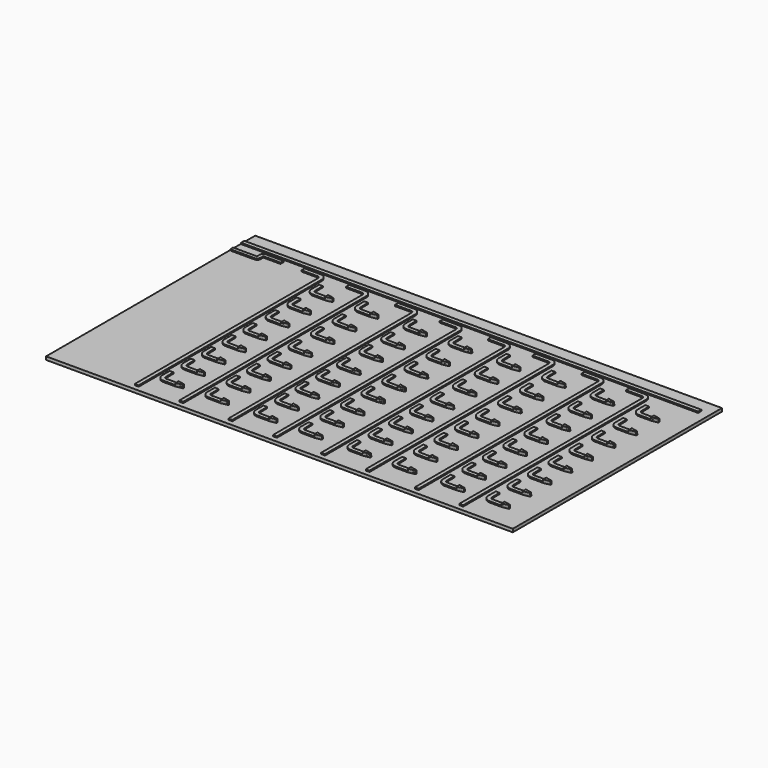
from build123d import *

# Parameters (mm, degrees)
F0_W     = 3719.7125814855
F0_H     = 2083.3632275462
F1_DEPTH = 25.4
F3_DEPTH = 10.16
F5_DEPTH = 7.62
F7_DEPTH = 7.62
F9_DEPTH = 10.16
F8_W     = 3642.5955891609
F8_H     = 31.8665504456


# Not quite as in the source:
# - a feature names something its author has since deleted; it is built from what else it names


with BuildPart() as f1:
    # F0 (on Top) → F1 (new body)
    with BuildSketch(Plane.XY):
        with Locations((924.2976289243, 427.4040535092)):
            Rectangle(F0_W, F0_H)
    extrude(amount=-F1_DEPTH)


with BuildPart() as f3:
    # F2 (on face) → F3 (new body)
    with BuildSketch(Plane.XY):
        with BuildLine():
            Line((0, 4.8675285652), (-51.4132715762, 16.0222817212))
            Line((-51.4132715762, 16.0222817212), (-149.2118090391, 16.0222817212))
            ThreePointArc((-149.2118090391, 16.0222817212), (-163.1179000848, 21.7124932059), (-169.0462678671, 35.5187356472))
            Line((-169.0462678671, 35.5187356472), (-170.3702134564, 112.54149833))
            Line((-170.3702134564, 112.54149833), (-199.8733133078, 112.0343690405))
            Line((-199.8733133078, 112.0343690405), (-199.8733133078, 35.5187356472))
            ThreePointArc((-199.8733133078, 35.5187356472), (-184.8444308949, 0.045176502), (-149.2118090391, -14.602586627))
            Line((-149.2118090391, -14.602586627), (-51.4132715762, -14.602586627))
            Line((-51.4132715762, -14.602586627), (0, -4.8675285652))
            Line((0, -4.8675285652), (0, 4.8675285652))
        make_face()
        with BuildLine():
            Line((0, 210.3862510994), (-51.4132715762, 221.5410042554))
            Line((-51.4132715762, 221.5410042554), (-149.2118090391, 221.5410042554))
            ThreePointArc((-149.2118090391, 221.5410042554), (-163.1179000848, 227.23121574), (-169.0462678671, 241.0374581814))
            Line((-169.0462678671, 241.0374581814), (-170.3702134564, 318.0602208642))
            Line((-170.3702134564, 318.0602208642), (-199.8733133078, 317.5530915746))
            Line((-199.8733133078, 317.5530915746), (-199.8733133078, 241.0374581814))
            ThreePointArc((-199.8733133078, 241.0374581814), (-184.8444308949, 205.5638990362), (-149.2118090391, 190.9161359072))
            Line((-149.2118090391, 190.9161359072), (-51.4132715762, 190.9161359072))
            Line((-51.4132715762, 190.9161359072), (0, 200.651193969))
            Line((0, 200.651193969), (0, 210.3862510994))
        make_face()
        with BuildLine():
            Line((0, -198.6540211365), (-51.4132715762, -187.4992679805))
            Line((-51.4132715762, -187.4992679805), (-149.2118090391, -187.4992679805))
            ThreePointArc((-149.2118090391, -187.4992679805), (-163.1179000848, -181.8090564958), (-169.0462678671, -168.0028140545))
            Line((-169.0462678671, -168.0028140545), (-170.3702134564, -90.9800513717))
            Line((-170.3702134564, -90.9800513717), (-199.8733133078, -91.4871806612))
            Line((-199.8733133078, -91.4871806612), (-199.8733133078, -168.0028140545))
            ThreePointArc((-199.8733133078, -168.0028140545), (-184.8444308949, -203.4763731996), (-149.2118090391, -218.1241363287))
            Line((-149.2118090391, -218.1241363287), (-51.4132715762, -218.1241363287))
            Line((-51.4132715762, -218.1241363287), (0, -208.3890782669))
            Line((0, -208.3890782669), (0, -198.6540211365))
        make_face()
        with BuildLine():
            Line((0, -409.4740850851), (-51.4132715762, -398.3193319291))
            Line((-51.4132715762, -398.3193319291), (-149.2118090391, -398.3193319291))
            ThreePointArc((-149.2118090391, -398.3193319291), (-163.1179000848, -392.6291204445), (-169.0462678671, -378.8228780031))
            Line((-169.0462678671, -378.8228780031), (-170.3702134564, -301.8001153203))
            Line((-170.3702134564, -301.8001153203), (-199.8733133078, -302.3072446099))
            Line((-199.8733133078, -302.3072446099), (-199.8733133078, -378.8228780031))
            ThreePointArc((-199.8733133078, -378.8228780031), (-184.8444308949, -414.2964371483), (-149.2118090391, -428.9442002773))
            Line((-149.2118090391, -428.9442002773), (-51.4132715762, -428.9442002773))
            Line((-51.4132715762, -428.9442002773), (0, -419.2091422155))
            Line((0, -419.2091422155), (0, -409.4740850851))
        make_face()
        with BuildLine():
            Line((0, 418.081481941), (-51.4132715762, 429.2362350971))
            Line((-51.4132715762, 429.2362350971), (-149.2118090391, 429.2362350971))
            ThreePointArc((-149.2118090391, 429.2362350971), (-163.1179000848, 434.9264465817), (-169.0462678671, 448.732689023))
            Line((-169.0462678671, 448.732689023), (-170.3702134564, 525.7554517058))
            Line((-170.3702134564, 525.7554517058), (-199.8733133078, 525.2483224163))
            Line((-199.8733133078, 525.2483224163), (-199.8733133078, 448.732689023))
            ThreePointArc((-199.8733133078, 448.732689023), (-184.8444308949, 413.2591298779), (-149.2118090391, 398.6113667488))
            Line((-149.2118090391, 398.6113667488), (-51.4132715762, 398.6113667488))
            Line((-51.4132715762, 398.6113667488), (0, 408.3464248106))
            Line((0, 408.3464248106), (0, 418.081481941))
        make_face()
        with BuildLine():
            Line((0, 640.5441214507), (-51.4132715762, 651.6988746067))
            Line((-51.4132715762, 651.6988746067), (-149.2118090391, 651.6988746067))
            ThreePointArc((-149.2118090391, 651.6988746067), (-163.1179000848, 657.3890860913), (-169.0462678671, 671.1953285327))
            Line((-169.0462678671, 671.1953285327), (-170.3702134564, 748.2180912155))
            Line((-170.3702134564, 748.2180912155), (-199.8733133078, 747.7109619259))
            Line((-199.8733133078, 747.7109619259), (-199.8733133078, 671.1953285327))
            ThreePointArc((-199.8733133078, 671.1953285327), (-184.8444308949, 635.7217693875), (-149.2118090391, 621.0740062585))
            Line((-149.2118090391, 621.0740062585), (-51.4132715762, 621.0740062585))
            Line((-51.4132715762, 621.0740062585), (0, 630.8090643202))
            Line((0, 630.8090643202), (0, 640.5441214507))
        make_face()
        with BuildLine():
            Line((0, 857.8696446493), (-51.4132715762, 869.0243978053))
            Line((-51.4132715762, 869.0243978053), (-149.2118090391, 869.0243978053))
            ThreePointArc((-149.2118090391, 869.0243978053), (-163.1179000848, 874.71460929), (-169.0462678671, 888.5208517313))
            Line((-169.0462678671, 888.5208517313), (-170.3702134564, 965.5436144141))
            Line((-170.3702134564, 965.5436144141), (-199.8733133078, 965.0364851246))
            Line((-199.8733133078, 965.0364851246), (-199.8733133078, 888.5208517313))
            ThreePointArc((-199.8733133078, 888.5208517313), (-184.8444308949, 853.0472925861), (-149.2118090391, 838.3995294571))
            Line((-149.2118090391, 838.3995294571), (-51.4132715762, 838.3995294571))
            Line((-51.4132715762, 838.3995294571), (0, 848.1345875189))
            Line((0, 848.1345875189), (0, 857.8696446493))
        make_face()
        with BuildLine():
            Line((0, 1078.9936976507), (-51.4132715762, 1090.1484508067))
            Line((-51.4132715762, 1090.1484508067), (-149.2118090391, 1090.1484508067))
            ThreePointArc((-149.2118090391, 1090.1484508067), (-163.1179000848, 1095.8386622914), (-169.0462678671, 1109.6449047327))
            Line((-169.0462678671, 1109.6449047327), (-170.3702134564, 1186.6676674155))
            Line((-170.3702134564, 1186.6676674155), (-199.8733133078, 1186.160538126))
            Line((-199.8733133078, 1186.160538126), (-199.8733133078, 1109.6449047327))
            ThreePointArc((-199.8733133078, 1109.6449047327), (-184.8444308949, 1074.1713455875), (-149.2118090391, 1059.5235824585))
            Line((-149.2118090391, 1059.5235824585), (-51.4132715762, 1059.5235824585))
            Line((-51.4132715762, 1059.5235824585), (0, 1069.2586405203))
            Line((0, 1069.2586405203), (0, 1078.9936976507))
        make_face()
        with BuildLine():
            Line((360.0319474936, 4.8675285652), (308.6186759174, 16.0222817212))
            Line((308.6186759174, 16.0222817212), (210.8201384544, 16.0222817212))
            ThreePointArc((210.8201384544, 16.0222817212), (196.9140474087, 21.7124932059), (190.9856796265, 35.5187356472))
            Line((190.9856796265, 35.5187356472), (189.6617340371, 112.54149833))
            Line((189.6617340371, 112.54149833), (160.1586341858, 112.0343690405))
            Line((160.1586341858, 112.0343690405), (160.1586341858, 35.5187356472))
            ThreePointArc((160.1586341858, 35.5187356472), (175.1875165986, 0.045176502), (210.8201384544, -14.602586627))
            Line((210.8201384544, -14.602586627), (308.6186759174, -14.602586627))
            Line((308.6186759174, -14.602586627), (360.0319474936, -4.8675285652))
            Line((360.0319474936, -4.8675285652), (360.0319474936, 4.8675285652))
        make_face()
        with BuildLine():
            Line((360.0319474936, 210.3862510994), (308.6186759174, 221.5410042554))
            Line((308.6186759174, 221.5410042554), (210.8201384544, 221.5410042554))
            ThreePointArc((210.8201384544, 221.5410042554), (196.9140474087, 227.23121574), (190.9856796265, 241.0374581814))
            Line((190.9856796265, 241.0374581814), (189.6617340371, 318.0602208642))
            Line((189.6617340371, 318.0602208642), (160.1586341858, 317.5530915746))
            Line((160.1586341858, 317.5530915746), (160.1586341858, 241.0374581814))
            ThreePointArc((160.1586341858, 241.0374581814), (175.1875165986, 205.5638990362), (210.8201384544, 190.9161359072))
            Line((210.8201384544, 190.9161359072), (308.6186759174, 190.9161359072))
            Line((308.6186759174, 190.9161359072), (360.0319474936, 200.651193969))
            Line((360.0319474936, 200.651193969), (360.0319474936, 210.3862510994))
        make_face()
        with BuildLine():
            Line((360.0319474936, -198.6540211365), (308.6186759174, -187.4992679805))
            Line((308.6186759174, -187.4992679805), (210.8201384544, -187.4992679805))
            ThreePointArc((210.8201384544, -187.4992679805), (196.9140474087, -181.8090564958), (190.9856796265, -168.0028140545))
            Line((190.9856796265, -168.0028140545), (189.6617340371, -90.9800513717))
            Line((189.6617340371, -90.9800513717), (160.1586341858, -91.4871806612))
            Line((160.1586341858, -91.4871806612), (160.1586341858, -168.0028140545))
            ThreePointArc((160.1586341858, -168.0028140545), (175.1875165986, -203.4763731996), (210.8201384544, -218.1241363287))
            Line((210.8201384544, -218.1241363287), (308.6186759174, -218.1241363287))
            Line((308.6186759174, -218.1241363287), (360.0319474936, -208.3890782669))
            Line((360.0319474936, -208.3890782669), (360.0319474936, -198.6540211365))
        make_face()
        with BuildLine():
            Line((360.0319474936, -409.4740850851), (308.6186759174, -398.3193319291))
            Line((308.6186759174, -398.3193319291), (210.8201384544, -398.3193319291))
            ThreePointArc((210.8201384544, -398.3193319291), (196.9140474087, -392.6291204445), (190.9856796265, -378.8228780031))
            Line((190.9856796265, -378.8228780031), (189.6617340371, -301.8001153203))
            Line((189.6617340371, -301.8001153203), (160.1586341858, -302.3072446099))
            Line((160.1586341858, -302.3072446099), (160.1586341858, -378.8228780031))
            ThreePointArc((160.1586341858, -378.8228780031), (175.1875165986, -414.2964371483), (210.8201384544, -428.9442002773))
            Line((210.8201384544, -428.9442002773), (308.6186759174, -428.9442002773))
            Line((308.6186759174, -428.9442002773), (360.0319474936, -419.2091422155))
            Line((360.0319474936, -419.2091422155), (360.0319474936, -409.4740850851))
        make_face()
        with BuildLine():
            Line((360.0319474936, 418.081481941), (308.6186759174, 429.2362350971))
            Line((308.6186759174, 429.2362350971), (210.8201384544, 429.2362350971))
            ThreePointArc((210.8201384544, 429.2362350971), (196.9140474087, 434.9264465817), (190.9856796265, 448.732689023))
            Line((190.9856796265, 448.732689023), (189.6617340371, 525.7554517058))
            Line((189.6617340371, 525.7554517058), (160.1586341858, 525.2483224163))
            Line((160.1586341858, 525.2483224163), (160.1586341858, 448.732689023))
            ThreePointArc((160.1586341858, 448.732689023), (175.1875165986, 413.2591298779), (210.8201384544, 398.6113667488))
            Line((210.8201384544, 398.6113667488), (308.6186759174, 398.6113667488))
            Line((308.6186759174, 398.6113667488), (360.0319474936, 408.3464248106))
            Line((360.0319474936, 408.3464248106), (360.0319474936, 418.081481941))
        make_face()
        with BuildLine():
            Line((360.0319474936, 640.5441214507), (308.6186759174, 651.6988746067))
            Line((308.6186759174, 651.6988746067), (210.8201384544, 651.6988746067))
            ThreePointArc((210.8201384544, 651.6988746067), (196.9140474087, 657.3890860913), (190.9856796265, 671.1953285327))
            Line((190.9856796265, 671.1953285327), (189.6617340371, 748.2180912155))
            Line((189.6617340371, 748.2180912155), (160.1586341858, 747.7109619259))
            Line((160.1586341858, 747.7109619259), (160.1586341858, 671.1953285327))
            ThreePointArc((160.1586341858, 671.1953285327), (175.1875165986, 635.7217693875), (210.8201384544, 621.0740062585))
            Line((210.8201384544, 621.0740062585), (308.6186759174, 621.0740062585))
            Line((308.6186759174, 621.0740062585), (360.0319474936, 630.8090643202))
            Line((360.0319474936, 630.8090643202), (360.0319474936, 640.5441214507))
        make_face()
        with BuildLine():
            Line((360.0319474936, 857.8696446493), (308.6186759174, 869.0243978053))
            Line((308.6186759174, 869.0243978053), (210.8201384544, 869.0243978053))
            ThreePointArc((210.8201384544, 869.0243978053), (196.9140474087, 874.71460929), (190.9856796265, 888.5208517313))
            Line((190.9856796265, 888.5208517313), (189.6617340371, 965.5436144141))
            Line((189.6617340371, 965.5436144141), (160.1586341858, 965.0364851246))
            Line((160.1586341858, 965.0364851246), (160.1586341858, 888.5208517313))
            ThreePointArc((160.1586341858, 888.5208517313), (175.1875165986, 853.0472925861), (210.8201384544, 838.3995294571))
            Line((210.8201384544, 838.3995294571), (308.6186759174, 838.3995294571))
            Line((308.6186759174, 838.3995294571), (360.0319474936, 848.1345875189))
            Line((360.0319474936, 848.1345875189), (360.0319474936, 857.8696446493))
        make_face()
        with BuildLine():
            Line((360.0319474936, 1078.9936976507), (308.6186759174, 1090.1484508067))
            Line((308.6186759174, 1090.1484508067), (210.8201384544, 1090.1484508067))
            ThreePointArc((210.8201384544, 1090.1484508067), (196.9140474087, 1095.8386622914), (190.9856796265, 1109.6449047327))
            Line((190.9856796265, 1109.6449047327), (189.6617340371, 1186.6676674155))
            Line((189.6617340371, 1186.6676674155), (160.1586341858, 1186.160538126))
            Line((160.1586341858, 1186.160538126), (160.1586341858, 1109.6449047327))
            ThreePointArc((160.1586341858, 1109.6449047327), (175.1875165986, 1074.1713455875), (210.8201384544, 1059.5235824585))
            Line((210.8201384544, 1059.5235824585), (308.6186759174, 1059.5235824585))
            Line((308.6186759174, 1059.5235824585), (360.0319474936, 1069.2586405203))
            Line((360.0319474936, 1069.2586405203), (360.0319474936, 1078.9936976507))
        make_face()
        with BuildLine():
            Line((746.7512339354, 4.8675285652), (695.3379623592, 16.0222817212))
            Line((695.3379623592, 16.0222817212), (597.5394248962, 16.0222817212))
            ThreePointArc((597.5394248962, 16.0222817212), (583.6333338505, 21.7124932059), (577.7049660683, 35.5187356472))
            Line((577.7049660683, 35.5187356472), (576.3810204789, 112.54149833))
            Line((576.3810204789, 112.54149833), (546.8779206276, 112.0343690405))
            Line((546.8779206276, 112.0343690405), (546.8779206276, 35.5187356472))
            ThreePointArc((546.8779206276, 35.5187356472), (561.9068030404, 0.045176502), (597.5394248962, -14.602586627))
            Line((597.5394248962, -14.602586627), (695.3379623592, -14.602586627))
            Line((695.3379623592, -14.602586627), (746.7512339354, -4.8675285652))
            Line((746.7512339354, -4.8675285652), (746.7512339354, 4.8675285652))
        make_face()
        with BuildLine():
            Line((746.7512339354, 210.3862510994), (695.3379623592, 221.5410042554))
            Line((695.3379623592, 221.5410042554), (597.5394248962, 221.5410042554))
            ThreePointArc((597.5394248962, 221.5410042554), (583.6333338505, 227.23121574), (577.7049660683, 241.0374581814))
            Line((577.7049660683, 241.0374581814), (576.3810204789, 318.0602208642))
            Line((576.3810204789, 318.0602208642), (546.8779206276, 317.5530915746))
            Line((546.8779206276, 317.5530915746), (546.8779206276, 241.0374581814))
            ThreePointArc((546.8779206276, 241.0374581814), (561.9068030404, 205.5638990362), (597.5394248962, 190.9161359072))
            Line((597.5394248962, 190.9161359072), (695.3379623592, 190.9161359072))
            Line((695.3379623592, 190.9161359072), (746.7512339354, 200.651193969))
            Line((746.7512339354, 200.651193969), (746.7512339354, 210.3862510994))
        make_face()
        with BuildLine():
            Line((746.7512339354, -198.6540211365), (695.3379623592, -187.4992679805))
            Line((695.3379623592, -187.4992679805), (597.5394248962, -187.4992679805))
            ThreePointArc((597.5394248962, -187.4992679805), (583.6333338505, -181.8090564958), (577.7049660683, -168.0028140545))
            Line((577.7049660683, -168.0028140545), (576.3810204789, -90.9800513717))
            Line((576.3810204789, -90.9800513717), (546.8779206276, -91.4871806612))
            Line((546.8779206276, -91.4871806612), (546.8779206276, -168.0028140545))
            ThreePointArc((546.8779206276, -168.0028140545), (561.9068030404, -203.4763731996), (597.5394248962, -218.1241363287))
            Line((597.5394248962, -218.1241363287), (695.3379623592, -218.1241363287))
            Line((695.3379623592, -218.1241363287), (746.7512339354, -208.3890782669))
            Line((746.7512339354, -208.3890782669), (746.7512339354, -198.6540211365))
        make_face()
        with BuildLine():
            Line((746.7512339354, -409.4740850851), (695.3379623592, -398.3193319291))
            Line((695.3379623592, -398.3193319291), (597.5394248962, -398.3193319291))
            ThreePointArc((597.5394248962, -398.3193319291), (583.6333338505, -392.6291204445), (577.7049660683, -378.8228780031))
            Line((577.7049660683, -378.8228780031), (576.3810204789, -301.8001153203))
            Line((576.3810204789, -301.8001153203), (546.8779206276, -302.3072446099))
            Line((546.8779206276, -302.3072446099), (546.8779206276, -378.8228780031))
            ThreePointArc((546.8779206276, -378.8228780031), (561.9068030404, -414.2964371483), (597.5394248962, -428.9442002773))
            Line((597.5394248962, -428.9442002773), (695.3379623592, -428.9442002773))
            Line((695.3379623592, -428.9442002773), (746.7512339354, -419.2091422155))
            Line((746.7512339354, -419.2091422155), (746.7512339354, -409.4740850851))
        make_face()
        with BuildLine():
            Line((746.7512339354, 418.081481941), (695.3379623592, 429.2362350971))
            Line((695.3379623592, 429.2362350971), (597.5394248962, 429.2362350971))
            ThreePointArc((597.5394248962, 429.2362350971), (583.6333338505, 434.9264465817), (577.7049660683, 448.732689023))
            Line((577.7049660683, 448.732689023), (576.3810204789, 525.7554517058))
            Line((576.3810204789, 525.7554517058), (546.8779206276, 525.2483224163))
            Line((546.8779206276, 525.2483224163), (546.8779206276, 448.732689023))
            ThreePointArc((546.8779206276, 448.732689023), (561.9068030404, 413.2591298779), (597.5394248962, 398.6113667488))
            Line((597.5394248962, 398.6113667488), (695.3379623592, 398.6113667488))
            Line((695.3379623592, 398.6113667488), (746.7512339354, 408.3464248106))
            Line((746.7512339354, 408.3464248106), (746.7512339354, 418.081481941))
        make_face()
        with BuildLine():
            Line((746.7512339354, 640.5441214507), (695.3379623592, 651.6988746067))
            Line((695.3379623592, 651.6988746067), (597.5394248962, 651.6988746067))
            ThreePointArc((597.5394248962, 651.6988746067), (583.6333338505, 657.3890860913), (577.7049660683, 671.1953285327))
            Line((577.7049660683, 671.1953285327), (576.3810204789, 748.2180912155))
            Line((576.3810204789, 748.2180912155), (546.8779206276, 747.7109619259))
            Line((546.8779206276, 747.7109619259), (546.8779206276, 671.1953285327))
            ThreePointArc((546.8779206276, 671.1953285327), (561.9068030404, 635.7217693875), (597.5394248962, 621.0740062585))
            Line((597.5394248962, 621.0740062585), (695.3379623592, 621.0740062585))
            Line((695.3379623592, 621.0740062585), (746.7512339354, 630.8090643202))
            Line((746.7512339354, 630.8090643202), (746.7512339354, 640.5441214507))
        make_face()
        with BuildLine():
            Line((746.7512339354, 857.8696446493), (695.3379623592, 869.0243978053))
            Line((695.3379623592, 869.0243978053), (597.5394248962, 869.0243978053))
            ThreePointArc((597.5394248962, 869.0243978053), (583.6333338505, 874.71460929), (577.7049660683, 888.5208517313))
            Line((577.7049660683, 888.5208517313), (576.3810204789, 965.5436144141))
            Line((576.3810204789, 965.5436144141), (546.8779206276, 965.0364851246))
            Line((546.8779206276, 965.0364851246), (546.8779206276, 888.5208517313))
            ThreePointArc((546.8779206276, 888.5208517313), (561.9068030404, 853.0472925861), (597.5394248962, 838.3995294571))
            Line((597.5394248962, 838.3995294571), (695.3379623592, 838.3995294571))
            Line((695.3379623592, 838.3995294571), (746.7512339354, 848.1345875189))
            Line((746.7512339354, 848.1345875189), (746.7512339354, 857.8696446493))
        make_face()
        with BuildLine():
            Line((746.7512339354, 1078.9936976507), (695.3379623592, 1090.1484508067))
            Line((695.3379623592, 1090.1484508067), (597.5394248962, 1090.1484508067))
            ThreePointArc((597.5394248962, 1090.1484508067), (583.6333338505, 1095.8386622914), (577.7049660683, 1109.6449047327))
            Line((577.7049660683, 1109.6449047327), (576.3810204789, 1186.6676674155))
            Line((576.3810204789, 1186.6676674155), (546.8779206276, 1186.160538126))
            Line((546.8779206276, 1186.160538126), (546.8779206276, 1109.6449047327))
            ThreePointArc((546.8779206276, 1109.6449047327), (561.9068030404, 1074.1713455875), (597.5394248962, 1059.5235824585))
            Line((597.5394248962, 1059.5235824585), (695.3379623592, 1059.5235824585))
            Line((695.3379623592, 1059.5235824585), (746.7512339354, 1069.2586405203))
            Line((746.7512339354, 1069.2586405203), (746.7512339354, 1078.9936976507))
        make_face()
        with BuildLine():
            Line((1106.7831814289, 4.8675285652), (1055.3699098527, 16.0222817212))
            Line((1055.3699098527, 16.0222817212), (957.5713723898, 16.0222817212))
            ThreePointArc((957.5713723898, 16.0222817212), (943.6652813441, 21.7124932059), (937.7369135618, 35.5187356472))
            Line((937.7369135618, 35.5187356472), (936.4129679725, 112.54149833))
            Line((936.4129679725, 112.54149833), (906.9098681211, 112.0343690405))
            Line((906.9098681211, 112.0343690405), (906.9098681211, 35.5187356472))
            ThreePointArc((906.9098681211, 35.5187356472), (921.938750534, 0.045176502), (957.5713723898, -14.602586627))
            Line((957.5713723898, -14.602586627), (1055.3699098527, -14.602586627))
            Line((1055.3699098527, -14.602586627), (1106.7831814289, -4.8675285652))
            Line((1106.7831814289, -4.8675285652), (1106.7831814289, 4.8675285652))
        make_face()
        with BuildLine():
            Line((1106.7831814289, 210.3862510994), (1055.3699098527, 221.5410042554))
            Line((1055.3699098527, 221.5410042554), (957.5713723898, 221.5410042554))
            ThreePointArc((957.5713723898, 221.5410042554), (943.6652813441, 227.23121574), (937.7369135618, 241.0374581814))
            Line((937.7369135618, 241.0374581814), (936.4129679725, 318.0602208642))
            Line((936.4129679725, 318.0602208642), (906.9098681211, 317.5530915746))
            Line((906.9098681211, 317.5530915746), (906.9098681211, 241.0374581814))
            ThreePointArc((906.9098681211, 241.0374581814), (921.938750534, 205.5638990362), (957.5713723898, 190.9161359072))
            Line((957.5713723898, 190.9161359072), (1055.3699098527, 190.9161359072))
            Line((1055.3699098527, 190.9161359072), (1106.7831814289, 200.651193969))
            Line((1106.7831814289, 200.651193969), (1106.7831814289, 210.3862510994))
        make_face()
        with BuildLine():
            Line((1106.7831814289, -198.6540211365), (1055.3699098527, -187.4992679805))
            Line((1055.3699098527, -187.4992679805), (957.5713723898, -187.4992679805))
            ThreePointArc((957.5713723898, -187.4992679805), (943.6652813441, -181.8090564958), (937.7369135618, -168.0028140545))
            Line((937.7369135618, -168.0028140545), (936.4129679725, -90.9800513717))
            Line((936.4129679725, -90.9800513717), (906.9098681211, -91.4871806612))
            Line((906.9098681211, -91.4871806612), (906.9098681211, -168.0028140545))
            ThreePointArc((906.9098681211, -168.0028140545), (921.938750534, -203.4763731996), (957.5713723898, -218.1241363287))
            Line((957.5713723898, -218.1241363287), (1055.3699098527, -218.1241363287))
            Line((1055.3699098527, -218.1241363287), (1106.7831814289, -208.3890782669))
            Line((1106.7831814289, -208.3890782669), (1106.7831814289, -198.6540211365))
        make_face()
        with BuildLine():
            Line((1106.7831814289, -409.4740850851), (1055.3699098527, -398.3193319291))
            Line((1055.3699098527, -398.3193319291), (957.5713723898, -398.3193319291))
            ThreePointArc((957.5713723898, -398.3193319291), (943.6652813441, -392.6291204445), (937.7369135618, -378.8228780031))
            Line((937.7369135618, -378.8228780031), (936.4129679725, -301.8001153203))
            Line((936.4129679725, -301.8001153203), (906.9098681211, -302.3072446099))
            Line((906.9098681211, -302.3072446099), (906.9098681211, -378.8228780031))
            ThreePointArc((906.9098681211, -378.8228780031), (921.938750534, -414.2964371483), (957.5713723898, -428.9442002773))
            Line((957.5713723898, -428.9442002773), (1055.3699098527, -428.9442002773))
            Line((1055.3699098527, -428.9442002773), (1106.7831814289, -419.2091422155))
            Line((1106.7831814289, -419.2091422155), (1106.7831814289, -409.4740850851))
        make_face()
        with BuildLine():
            Line((1106.7831814289, 418.081481941), (1055.3699098527, 429.2362350971))
            Line((1055.3699098527, 429.2362350971), (957.5713723898, 429.2362350971))
            ThreePointArc((957.5713723898, 429.2362350971), (943.6652813441, 434.9264465817), (937.7369135618, 448.732689023))
            Line((937.7369135618, 448.732689023), (936.4129679725, 525.7554517058))
            Line((936.4129679725, 525.7554517058), (906.9098681211, 525.2483224163))
            Line((906.9098681211, 525.2483224163), (906.9098681211, 448.732689023))
            ThreePointArc((906.9098681211, 448.732689023), (921.938750534, 413.2591298779), (957.5713723898, 398.6113667488))
            Line((957.5713723898, 398.6113667488), (1055.3699098527, 398.6113667488))
            Line((1055.3699098527, 398.6113667488), (1106.7831814289, 408.3464248106))
            Line((1106.7831814289, 408.3464248106), (1106.7831814289, 418.081481941))
        make_face()
        with BuildLine():
            Line((1106.7831814289, 640.5441214507), (1055.3699098527, 651.6988746067))
            Line((1055.3699098527, 651.6988746067), (957.5713723898, 651.6988746067))
            ThreePointArc((957.5713723898, 651.6988746067), (943.6652813441, 657.3890860913), (937.7369135618, 671.1953285327))
            Line((937.7369135618, 671.1953285327), (936.4129679725, 748.2180912155))
            Line((936.4129679725, 748.2180912155), (906.9098681211, 747.7109619259))
            Line((906.9098681211, 747.7109619259), (906.9098681211, 671.1953285327))
            ThreePointArc((906.9098681211, 671.1953285327), (921.938750534, 635.7217693875), (957.5713723898, 621.0740062585))
            Line((957.5713723898, 621.0740062585), (1055.3699098527, 621.0740062585))
            Line((1055.3699098527, 621.0740062585), (1106.7831814289, 630.8090643202))
            Line((1106.7831814289, 630.8090643202), (1106.7831814289, 640.5441214507))
        make_face()
        with BuildLine():
            Line((1106.7831814289, 857.8696446493), (1055.3699098527, 869.0243978053))
            Line((1055.3699098527, 869.0243978053), (957.5713723898, 869.0243978053))
            ThreePointArc((957.5713723898, 869.0243978053), (943.6652813441, 874.71460929), (937.7369135618, 888.5208517313))
            Line((937.7369135618, 888.5208517313), (936.4129679725, 965.5436144141))
            Line((936.4129679725, 965.5436144141), (906.9098681211, 965.0364851246))
            Line((906.9098681211, 965.0364851246), (906.9098681211, 888.5208517313))
            ThreePointArc((906.9098681211, 888.5208517313), (921.938750534, 853.0472925861), (957.5713723898, 838.3995294571))
            Line((957.5713723898, 838.3995294571), (1055.3699098527, 838.3995294571))
            Line((1055.3699098527, 838.3995294571), (1106.7831814289, 848.1345875189))
            Line((1106.7831814289, 848.1345875189), (1106.7831814289, 857.8696446493))
        make_face()
        with BuildLine():
            Line((1106.7831814289, 1078.9936976507), (1055.3699098527, 1090.1484508067))
            Line((1055.3699098527, 1090.1484508067), (957.5713723898, 1090.1484508067))
            ThreePointArc((957.5713723898, 1090.1484508067), (943.6652813441, 1095.8386622914), (937.7369135618, 1109.6449047327))
            Line((937.7369135618, 1109.6449047327), (936.4129679725, 1186.6676674155))
            Line((936.4129679725, 1186.6676674155), (906.9098681211, 1186.160538126))
            Line((906.9098681211, 1186.160538126), (906.9098681211, 1109.6449047327))
            ThreePointArc((906.9098681211, 1109.6449047327), (921.938750534, 1074.1713455875), (957.5713723898, 1059.5235824585))
            Line((957.5713723898, 1059.5235824585), (1055.3699098527, 1059.5235824585))
            Line((1055.3699098527, 1059.5235824585), (1106.7831814289, 1069.2586405203))
            Line((1106.7831814289, 1069.2586405203), (1106.7831814289, 1078.9936976507))
        make_face()
        with BuildLine():
            Line((1492.2146052122, 4.8675285652), (1440.801333636, 16.0222817212))
            Line((1440.801333636, 16.0222817212), (1343.0027961731, 16.0222817212))
            ThreePointArc((1343.0027961731, 16.0222817212), (1329.0967051274, 21.7124932059), (1323.1683373451, 35.5187356472))
            Line((1323.1683373451, 35.5187356472), (1321.8443917558, 112.54149833))
            Line((1321.8443917558, 112.54149833), (1292.3412919044, 112.0343690405))
            Line((1292.3412919044, 112.0343690405), (1292.3412919044, 35.5187356472))
            ThreePointArc((1292.3412919044, 35.5187356472), (1307.3701743173, 0.045176502), (1343.0027961731, -14.602586627))
            Line((1343.0027961731, -14.602586627), (1440.801333636, -14.602586627))
            Line((1440.801333636, -14.602586627), (1492.2146052122, -4.8675285652))
            Line((1492.2146052122, -4.8675285652), (1492.2146052122, 4.8675285652))
        make_face()
        with BuildLine():
            Line((1492.2146052122, 210.3862510994), (1440.801333636, 221.5410042554))
            Line((1440.801333636, 221.5410042554), (1343.0027961731, 221.5410042554))
            ThreePointArc((1343.0027961731, 221.5410042554), (1329.0967051274, 227.23121574), (1323.1683373451, 241.0374581814))
            Line((1323.1683373451, 241.0374581814), (1321.8443917558, 318.0602208642))
            Line((1321.8443917558, 318.0602208642), (1292.3412919044, 317.5530915746))
            Line((1292.3412919044, 317.5530915746), (1292.3412919044, 241.0374581814))
            ThreePointArc((1292.3412919044, 241.0374581814), (1307.3701743173, 205.5638990362), (1343.0027961731, 190.9161359072))
            Line((1343.0027961731, 190.9161359072), (1440.801333636, 190.9161359072))
            Line((1440.801333636, 190.9161359072), (1492.2146052122, 200.651193969))
            Line((1492.2146052122, 200.651193969), (1492.2146052122, 210.3862510994))
        make_face()
        with BuildLine():
            Line((1492.2146052122, -198.6540211365), (1440.801333636, -187.4992679805))
            Line((1440.801333636, -187.4992679805), (1343.0027961731, -187.4992679805))
            ThreePointArc((1343.0027961731, -187.4992679805), (1329.0967051274, -181.8090564958), (1323.1683373451, -168.0028140545))
            Line((1323.1683373451, -168.0028140545), (1321.8443917558, -90.9800513717))
            Line((1321.8443917558, -90.9800513717), (1292.3412919044, -91.4871806612))
            Line((1292.3412919044, -91.4871806612), (1292.3412919044, -168.0028140545))
            ThreePointArc((1292.3412919044, -168.0028140545), (1307.3701743173, -203.4763731996), (1343.0027961731, -218.1241363287))
            Line((1343.0027961731, -218.1241363287), (1440.801333636, -218.1241363287))
            Line((1440.801333636, -218.1241363287), (1492.2146052122, -208.3890782669))
            Line((1492.2146052122, -208.3890782669), (1492.2146052122, -198.6540211365))
        make_face()
        with BuildLine():
            Line((1492.2146052122, -409.4740850851), (1440.801333636, -398.3193319291))
            Line((1440.801333636, -398.3193319291), (1343.0027961731, -398.3193319291))
            ThreePointArc((1343.0027961731, -398.3193319291), (1329.0967051274, -392.6291204445), (1323.1683373451, -378.8228780031))
            Line((1323.1683373451, -378.8228780031), (1321.8443917558, -301.8001153203))
            Line((1321.8443917558, -301.8001153203), (1292.3412919044, -302.3072446099))
            Line((1292.3412919044, -302.3072446099), (1292.3412919044, -378.8228780031))
            ThreePointArc((1292.3412919044, -378.8228780031), (1307.3701743173, -414.2964371483), (1343.0027961731, -428.9442002773))
            Line((1343.0027961731, -428.9442002773), (1440.801333636, -428.9442002773))
            Line((1440.801333636, -428.9442002773), (1492.2146052122, -419.2091422155))
            Line((1492.2146052122, -419.2091422155), (1492.2146052122, -409.4740850851))
        make_face()
        with BuildLine():
            Line((1492.2146052122, 418.081481941), (1440.801333636, 429.2362350971))
            Line((1440.801333636, 429.2362350971), (1343.0027961731, 429.2362350971))
            ThreePointArc((1343.0027961731, 429.2362350971), (1329.0967051274, 434.9264465817), (1323.1683373451, 448.732689023))
            Line((1323.1683373451, 448.732689023), (1321.8443917558, 525.7554517058))
            Line((1321.8443917558, 525.7554517058), (1292.3412919044, 525.2483224163))
            Line((1292.3412919044, 525.2483224163), (1292.3412919044, 448.732689023))
            ThreePointArc((1292.3412919044, 448.732689023), (1307.3701743173, 413.2591298779), (1343.0027961731, 398.6113667488))
            Line((1343.0027961731, 398.6113667488), (1440.801333636, 398.6113667488))
            Line((1440.801333636, 398.6113667488), (1492.2146052122, 408.3464248106))
            Line((1492.2146052122, 408.3464248106), (1492.2146052122, 418.081481941))
        make_face()
        with BuildLine():
            Line((1492.2146052122, 640.5441214507), (1440.801333636, 651.6988746067))
            Line((1440.801333636, 651.6988746067), (1343.0027961731, 651.6988746067))
            ThreePointArc((1343.0027961731, 651.6988746067), (1329.0967051274, 657.3890860913), (1323.1683373451, 671.1953285327))
            Line((1323.1683373451, 671.1953285327), (1321.8443917558, 748.2180912155))
            Line((1321.8443917558, 748.2180912155), (1292.3412919044, 747.7109619259))
            Line((1292.3412919044, 747.7109619259), (1292.3412919044, 671.1953285327))
            ThreePointArc((1292.3412919044, 671.1953285327), (1307.3701743173, 635.7217693875), (1343.0027961731, 621.0740062585))
            Line((1343.0027961731, 621.0740062585), (1440.801333636, 621.0740062585))
            Line((1440.801333636, 621.0740062585), (1492.2146052122, 630.8090643202))
            Line((1492.2146052122, 630.8090643202), (1492.2146052122, 640.5441214507))
        make_face()
        with BuildLine():
            Line((1492.2146052122, 857.8696446493), (1440.801333636, 869.0243978053))
            Line((1440.801333636, 869.0243978053), (1343.0027961731, 869.0243978053))
            ThreePointArc((1343.0027961731, 869.0243978053), (1329.0967051274, 874.71460929), (1323.1683373451, 888.5208517313))
            Line((1323.1683373451, 888.5208517313), (1321.8443917558, 965.5436144141))
            Line((1321.8443917558, 965.5436144141), (1292.3412919044, 965.0364851246))
            Line((1292.3412919044, 965.0364851246), (1292.3412919044, 888.5208517313))
            ThreePointArc((1292.3412919044, 888.5208517313), (1307.3701743173, 853.0472925861), (1343.0027961731, 838.3995294571))
            Line((1343.0027961731, 838.3995294571), (1440.801333636, 838.3995294571))
            Line((1440.801333636, 838.3995294571), (1492.2146052122, 848.1345875189))
            Line((1492.2146052122, 848.1345875189), (1492.2146052122, 857.8696446493))
        make_face()
        with BuildLine():
            Line((1492.2146052122, 1078.9936976507), (1440.801333636, 1090.1484508067))
            Line((1440.801333636, 1090.1484508067), (1343.0027961731, 1090.1484508067))
            ThreePointArc((1343.0027961731, 1090.1484508067), (1329.0967051274, 1095.8386622914), (1323.1683373451, 1109.6449047327))
            Line((1323.1683373451, 1109.6449047327), (1321.8443917558, 1186.6676674155))
            Line((1321.8443917558, 1186.6676674155), (1292.3412919044, 1186.160538126))
            Line((1292.3412919044, 1186.160538126), (1292.3412919044, 1109.6449047327))
            ThreePointArc((1292.3412919044, 1109.6449047327), (1307.3701743173, 1074.1713455875), (1343.0027961731, 1059.5235824585))
            Line((1343.0027961731, 1059.5235824585), (1440.801333636, 1059.5235824585))
            Line((1440.801333636, 1059.5235824585), (1492.2146052122, 1069.2586405203))
            Line((1492.2146052122, 1069.2586405203), (1492.2146052122, 1078.9936976507))
        make_face()
        with BuildLine():
            Line((1852.2465527058, 4.8675285652), (1800.8332811296, 16.0222817212))
            Line((1800.8332811296, 16.0222817212), (1703.0347436666, 16.0222817212))
            ThreePointArc((1703.0347436666, 16.0222817212), (1689.1286526209, 21.7124932059), (1683.2002848387, 35.5187356472))
            Line((1683.2002848387, 35.5187356472), (1681.8763392493, 112.54149833))
            Line((1681.8763392493, 112.54149833), (1652.373239398, 112.0343690405))
            Line((1652.373239398, 112.0343690405), (1652.373239398, 35.5187356472))
            ThreePointArc((1652.373239398, 35.5187356472), (1667.4021218108, 0.045176502), (1703.0347436666, -14.602586627))
            Line((1703.0347436666, -14.602586627), (1800.8332811296, -14.602586627))
            Line((1800.8332811296, -14.602586627), (1852.2465527058, -4.8675285652))
            Line((1852.2465527058, -4.8675285652), (1852.2465527058, 4.8675285652))
        make_face()
        with BuildLine():
            Line((1852.2465527058, 210.3862510994), (1800.8332811296, 221.5410042554))
            Line((1800.8332811296, 221.5410042554), (1703.0347436666, 221.5410042554))
            ThreePointArc((1703.0347436666, 221.5410042554), (1689.1286526209, 227.23121574), (1683.2002848387, 241.0374581814))
            Line((1683.2002848387, 241.0374581814), (1681.8763392493, 318.0602208642))
            Line((1681.8763392493, 318.0602208642), (1652.373239398, 317.5530915746))
            Line((1652.373239398, 317.5530915746), (1652.373239398, 241.0374581814))
            ThreePointArc((1652.373239398, 241.0374581814), (1667.4021218108, 205.5638990362), (1703.0347436666, 190.9161359072))
            Line((1703.0347436666, 190.9161359072), (1800.8332811296, 190.9161359072))
            Line((1800.8332811296, 190.9161359072), (1852.2465527058, 200.651193969))
            Line((1852.2465527058, 200.651193969), (1852.2465527058, 210.3862510994))
        make_face()
        with BuildLine():
            Line((1852.2465527058, -198.6540211365), (1800.8332811296, -187.4992679805))
            Line((1800.8332811296, -187.4992679805), (1703.0347436666, -187.4992679805))
            ThreePointArc((1703.0347436666, -187.4992679805), (1689.1286526209, -181.8090564958), (1683.2002848387, -168.0028140545))
            Line((1683.2002848387, -168.0028140545), (1681.8763392493, -90.9800513717))
            Line((1681.8763392493, -90.9800513717), (1652.373239398, -91.4871806612))
            Line((1652.373239398, -91.4871806612), (1652.373239398, -168.0028140545))
            ThreePointArc((1652.373239398, -168.0028140545), (1667.4021218108, -203.4763731996), (1703.0347436666, -218.1241363287))
            Line((1703.0347436666, -218.1241363287), (1800.8332811296, -218.1241363287))
            Line((1800.8332811296, -218.1241363287), (1852.2465527058, -208.3890782669))
            Line((1852.2465527058, -208.3890782669), (1852.2465527058, -198.6540211365))
        make_face()
        with BuildLine():
            Line((1852.2465527058, -409.4740850851), (1800.8332811296, -398.3193319291))
            Line((1800.8332811296, -398.3193319291), (1703.0347436666, -398.3193319291))
            ThreePointArc((1703.0347436666, -398.3193319291), (1689.1286526209, -392.6291204445), (1683.2002848387, -378.8228780031))
            Line((1683.2002848387, -378.8228780031), (1681.8763392493, -301.8001153203))
            Line((1681.8763392493, -301.8001153203), (1652.373239398, -302.3072446099))
            Line((1652.373239398, -302.3072446099), (1652.373239398, -378.8228780031))
            ThreePointArc((1652.373239398, -378.8228780031), (1667.4021218108, -414.2964371483), (1703.0347436666, -428.9442002773))
            Line((1703.0347436666, -428.9442002773), (1800.8332811296, -428.9442002773))
            Line((1800.8332811296, -428.9442002773), (1852.2465527058, -419.2091422155))
            Line((1852.2465527058, -419.2091422155), (1852.2465527058, -409.4740850851))
        make_face()
        with BuildLine():
            Line((1852.2465527058, 418.081481941), (1800.8332811296, 429.2362350971))
            Line((1800.8332811296, 429.2362350971), (1703.0347436666, 429.2362350971))
            ThreePointArc((1703.0347436666, 429.2362350971), (1689.1286526209, 434.9264465817), (1683.2002848387, 448.732689023))
            Line((1683.2002848387, 448.732689023), (1681.8763392493, 525.7554517058))
            Line((1681.8763392493, 525.7554517058), (1652.373239398, 525.2483224163))
            Line((1652.373239398, 525.2483224163), (1652.373239398, 448.732689023))
            ThreePointArc((1652.373239398, 448.732689023), (1667.4021218108, 413.2591298779), (1703.0347436666, 398.6113667488))
            Line((1703.0347436666, 398.6113667488), (1800.8332811296, 398.6113667488))
            Line((1800.8332811296, 398.6113667488), (1852.2465527058, 408.3464248106))
            Line((1852.2465527058, 408.3464248106), (1852.2465527058, 418.081481941))
        make_face()
        with BuildLine():
            Line((1852.2465527058, 640.5441214507), (1800.8332811296, 651.6988746067))
            Line((1800.8332811296, 651.6988746067), (1703.0347436666, 651.6988746067))
            ThreePointArc((1703.0347436666, 651.6988746067), (1689.1286526209, 657.3890860913), (1683.2002848387, 671.1953285327))
            Line((1683.2002848387, 671.1953285327), (1681.8763392493, 748.2180912155))
            Line((1681.8763392493, 748.2180912155), (1652.373239398, 747.7109619259))
            Line((1652.373239398, 747.7109619259), (1652.373239398, 671.1953285327))
            ThreePointArc((1652.373239398, 671.1953285327), (1667.4021218108, 635.7217693875), (1703.0347436666, 621.0740062585))
            Line((1703.0347436666, 621.0740062585), (1800.8332811296, 621.0740062585))
            Line((1800.8332811296, 621.0740062585), (1852.2465527058, 630.8090643202))
            Line((1852.2465527058, 630.8090643202), (1852.2465527058, 640.5441214507))
        make_face()
        with BuildLine():
            Line((1852.2465527058, 857.8696446493), (1800.8332811296, 869.0243978053))
            Line((1800.8332811296, 869.0243978053), (1703.0347436666, 869.0243978053))
            ThreePointArc((1703.0347436666, 869.0243978053), (1689.1286526209, 874.71460929), (1683.2002848387, 888.5208517313))
            Line((1683.2002848387, 888.5208517313), (1681.8763392493, 965.5436144141))
            Line((1681.8763392493, 965.5436144141), (1652.373239398, 965.0364851246))
            Line((1652.373239398, 965.0364851246), (1652.373239398, 888.5208517313))
            ThreePointArc((1652.373239398, 888.5208517313), (1667.4021218108, 853.0472925861), (1703.0347436666, 838.3995294571))
            Line((1703.0347436666, 838.3995294571), (1800.8332811296, 838.3995294571))
            Line((1800.8332811296, 838.3995294571), (1852.2465527058, 848.1345875189))
            Line((1852.2465527058, 848.1345875189), (1852.2465527058, 857.8696446493))
        make_face()
        with BuildLine():
            Line((1852.2465527058, 1078.9936976507), (1800.8332811296, 1090.1484508067))
            Line((1800.8332811296, 1090.1484508067), (1703.0347436666, 1090.1484508067))
            ThreePointArc((1703.0347436666, 1090.1484508067), (1689.1286526209, 1095.8386622914), (1683.2002848387, 1109.6449047327))
            Line((1683.2002848387, 1109.6449047327), (1681.8763392493, 1186.6676674155))
            Line((1681.8763392493, 1186.6676674155), (1652.373239398, 1186.160538126))
            Line((1652.373239398, 1186.160538126), (1652.373239398, 1109.6449047327))
            ThreePointArc((1652.373239398, 1109.6449047327), (1667.4021218108, 1074.1713455875), (1703.0347436666, 1059.5235824585))
            Line((1703.0347436666, 1059.5235824585), (1800.8332811296, 1059.5235824585))
            Line((1800.8332811296, 1059.5235824585), (1852.2465527058, 1069.2586405203))
            Line((1852.2465527058, 1069.2586405203), (1852.2465527058, 1078.9936976507))
        make_face()
        with BuildLine():
            Line((2238.9658391476, 4.8675285652), (2187.5525675714, 16.0222817212))
            Line((2187.5525675714, 16.0222817212), (2089.7540301085, 16.0222817212))
            ThreePointArc((2089.7540301085, 16.0222817212), (2075.8479390627, 21.7124932059), (2069.9195712805, 35.5187356472))
            Line((2069.9195712805, 35.5187356472), (2068.5956256911, 112.54149833))
            Line((2068.5956256911, 112.54149833), (2039.0925258398, 112.0343690405))
            Line((2039.0925258398, 112.0343690405), (2039.0925258398, 35.5187356472))
            ThreePointArc((2039.0925258398, 35.5187356472), (2054.1214082526, 0.045176502), (2089.7540301085, -14.602586627))
            Line((2089.7540301085, -14.602586627), (2187.5525675714, -14.602586627))
            Line((2187.5525675714, -14.602586627), (2238.9658391476, -4.8675285652))
            Line((2238.9658391476, -4.8675285652), (2238.9658391476, 4.8675285652))
        make_face()
        with BuildLine():
            Line((2238.9658391476, 210.3862510994), (2187.5525675714, 221.5410042554))
            Line((2187.5525675714, 221.5410042554), (2089.7540301085, 221.5410042554))
            ThreePointArc((2089.7540301085, 221.5410042554), (2075.8479390627, 227.23121574), (2069.9195712805, 241.0374581814))
            Line((2069.9195712805, 241.0374581814), (2068.5956256911, 318.0602208642))
            Line((2068.5956256911, 318.0602208642), (2039.0925258398, 317.5530915746))
            Line((2039.0925258398, 317.5530915746), (2039.0925258398, 241.0374581814))
            ThreePointArc((2039.0925258398, 241.0374581814), (2054.1214082526, 205.5638990362), (2089.7540301085, 190.9161359072))
            Line((2089.7540301085, 190.9161359072), (2187.5525675714, 190.9161359072))
            Line((2187.5525675714, 190.9161359072), (2238.9658391476, 200.651193969))
            Line((2238.9658391476, 200.651193969), (2238.9658391476, 210.3862510994))
        make_face()
        with BuildLine():
            Line((2238.9658391476, -198.6540211365), (2187.5525675714, -187.4992679805))
            Line((2187.5525675714, -187.4992679805), (2089.7540301085, -187.4992679805))
            ThreePointArc((2089.7540301085, -187.4992679805), (2075.8479390627, -181.8090564958), (2069.9195712805, -168.0028140545))
            Line((2069.9195712805, -168.0028140545), (2068.5956256911, -90.9800513717))
            Line((2068.5956256911, -90.9800513717), (2039.0925258398, -91.4871806612))
            Line((2039.0925258398, -91.4871806612), (2039.0925258398, -168.0028140545))
            ThreePointArc((2039.0925258398, -168.0028140545), (2054.1214082526, -203.4763731996), (2089.7540301085, -218.1241363287))
            Line((2089.7540301085, -218.1241363287), (2187.5525675714, -218.1241363287))
            Line((2187.5525675714, -218.1241363287), (2238.9658391476, -208.3890782669))
            Line((2238.9658391476, -208.3890782669), (2238.9658391476, -198.6540211365))
        make_face()
        with BuildLine():
            Line((2238.9658391476, -409.4740850851), (2187.5525675714, -398.3193319291))
            Line((2187.5525675714, -398.3193319291), (2089.7540301085, -398.3193319291))
            ThreePointArc((2089.7540301085, -398.3193319291), (2075.8479390627, -392.6291204445), (2069.9195712805, -378.8228780031))
            Line((2069.9195712805, -378.8228780031), (2068.5956256911, -301.8001153203))
            Line((2068.5956256911, -301.8001153203), (2039.0925258398, -302.3072446099))
            Line((2039.0925258398, -302.3072446099), (2039.0925258398, -378.8228780031))
            ThreePointArc((2039.0925258398, -378.8228780031), (2054.1214082526, -414.2964371483), (2089.7540301085, -428.9442002773))
            Line((2089.7540301085, -428.9442002773), (2187.5525675714, -428.9442002773))
            Line((2187.5525675714, -428.9442002773), (2238.9658391476, -419.2091422155))
            Line((2238.9658391476, -419.2091422155), (2238.9658391476, -409.4740850851))
        make_face()
        with BuildLine():
            Line((2238.9658391476, 418.081481941), (2187.5525675714, 429.2362350971))
            Line((2187.5525675714, 429.2362350971), (2089.7540301085, 429.2362350971))
            ThreePointArc((2089.7540301085, 429.2362350971), (2075.8479390627, 434.9264465817), (2069.9195712805, 448.732689023))
            Line((2069.9195712805, 448.732689023), (2068.5956256911, 525.7554517058))
            Line((2068.5956256911, 525.7554517058), (2039.0925258398, 525.2483224163))
            Line((2039.0925258398, 525.2483224163), (2039.0925258398, 448.732689023))
            ThreePointArc((2039.0925258398, 448.732689023), (2054.1214082526, 413.2591298779), (2089.7540301085, 398.6113667488))
            Line((2089.7540301085, 398.6113667488), (2187.5525675714, 398.6113667488))
            Line((2187.5525675714, 398.6113667488), (2238.9658391476, 408.3464248106))
            Line((2238.9658391476, 408.3464248106), (2238.9658391476, 418.081481941))
        make_face()
        with BuildLine():
            Line((2238.9658391476, 640.5441214507), (2187.5525675714, 651.6988746067))
            Line((2187.5525675714, 651.6988746067), (2089.7540301085, 651.6988746067))
            ThreePointArc((2089.7540301085, 651.6988746067), (2075.8479390627, 657.3890860913), (2069.9195712805, 671.1953285327))
            Line((2069.9195712805, 671.1953285327), (2068.5956256911, 748.2180912155))
            Line((2068.5956256911, 748.2180912155), (2039.0925258398, 747.7109619259))
            Line((2039.0925258398, 747.7109619259), (2039.0925258398, 671.1953285327))
            ThreePointArc((2039.0925258398, 671.1953285327), (2054.1214082526, 635.7217693875), (2089.7540301085, 621.0740062585))
            Line((2089.7540301085, 621.0740062585), (2187.5525675714, 621.0740062585))
            Line((2187.5525675714, 621.0740062585), (2238.9658391476, 630.8090643202))
            Line((2238.9658391476, 630.8090643202), (2238.9658391476, 640.5441214507))
        make_face()
        with BuildLine():
            Line((2238.9658391476, 857.8696446493), (2187.5525675714, 869.0243978053))
            Line((2187.5525675714, 869.0243978053), (2089.7540301085, 869.0243978053))
            ThreePointArc((2089.7540301085, 869.0243978053), (2075.8479390627, 874.71460929), (2069.9195712805, 888.5208517313))
            Line((2069.9195712805, 888.5208517313), (2068.5956256911, 965.5436144141))
            Line((2068.5956256911, 965.5436144141), (2039.0925258398, 965.0364851246))
            Line((2039.0925258398, 965.0364851246), (2039.0925258398, 888.5208517313))
            ThreePointArc((2039.0925258398, 888.5208517313), (2054.1214082526, 853.0472925861), (2089.7540301085, 838.3995294571))
            Line((2089.7540301085, 838.3995294571), (2187.5525675714, 838.3995294571))
            Line((2187.5525675714, 838.3995294571), (2238.9658391476, 848.1345875189))
            Line((2238.9658391476, 848.1345875189), (2238.9658391476, 857.8696446493))
        make_face()
        with BuildLine():
            Line((2238.9658391476, 1078.9936976507), (2187.5525675714, 1090.1484508067))
            Line((2187.5525675714, 1090.1484508067), (2089.7540301085, 1090.1484508067))
            ThreePointArc((2089.7540301085, 1090.1484508067), (2075.8479390627, 1095.8386622914), (2069.9195712805, 1109.6449047327))
            Line((2069.9195712805, 1109.6449047327), (2068.5956256911, 1186.6676674155))
            Line((2068.5956256911, 1186.6676674155), (2039.0925258398, 1186.160538126))
            Line((2039.0925258398, 1186.160538126), (2039.0925258398, 1109.6449047327))
            ThreePointArc((2039.0925258398, 1109.6449047327), (2054.1214082526, 1074.1713455875), (2089.7540301085, 1059.5235824585))
            Line((2089.7540301085, 1059.5235824585), (2187.5525675714, 1059.5235824585))
            Line((2187.5525675714, 1059.5235824585), (2238.9658391476, 1069.2586405203))
            Line((2238.9658391476, 1069.2586405203), (2238.9658391476, 1078.9936976507))
        make_face()
        with BuildLine():
            Line((2598.9977866411, 4.8675285652), (2547.584515065, 16.0222817212))
            Line((2547.584515065, 16.0222817212), (2449.785977602, 16.0222817212))
            ThreePointArc((2449.785977602, 16.0222817212), (2435.8798865563, 21.7124932059), (2429.951518774, 35.5187356472))
            Line((2429.951518774, 35.5187356472), (2428.6275731847, 112.54149833))
            Line((2428.6275731847, 112.54149833), (2399.1244733334, 112.0343690405))
            Line((2399.1244733334, 112.0343690405), (2399.1244733334, 35.5187356472))
            ThreePointArc((2399.1244733334, 35.5187356472), (2414.1533557462, 0.045176502), (2449.785977602, -14.602586627))
            Line((2449.785977602, -14.602586627), (2547.584515065, -14.602586627))
            Line((2547.584515065, -14.602586627), (2598.9977866411, -4.8675285652))
            Line((2598.9977866411, -4.8675285652), (2598.9977866411, 4.8675285652))
        make_face()
        with BuildLine():
            Line((2598.9977866411, 210.3862510994), (2547.584515065, 221.5410042554))
            Line((2547.584515065, 221.5410042554), (2449.785977602, 221.5410042554))
            ThreePointArc((2449.785977602, 221.5410042554), (2435.8798865563, 227.23121574), (2429.951518774, 241.0374581814))
            Line((2429.951518774, 241.0374581814), (2428.6275731847, 318.0602208642))
            Line((2428.6275731847, 318.0602208642), (2399.1244733334, 317.5530915746))
            Line((2399.1244733334, 317.5530915746), (2399.1244733334, 241.0374581814))
            ThreePointArc((2399.1244733334, 241.0374581814), (2414.1533557462, 205.5638990362), (2449.785977602, 190.9161359072))
            Line((2449.785977602, 190.9161359072), (2547.584515065, 190.9161359072))
            Line((2547.584515065, 190.9161359072), (2598.9977866411, 200.651193969))
            Line((2598.9977866411, 200.651193969), (2598.9977866411, 210.3862510994))
        make_face()
        with BuildLine():
            Line((2598.9977866411, -198.6540211365), (2547.584515065, -187.4992679805))
            Line((2547.584515065, -187.4992679805), (2449.785977602, -187.4992679805))
            ThreePointArc((2449.785977602, -187.4992679805), (2435.8798865563, -181.8090564958), (2429.951518774, -168.0028140545))
            Line((2429.951518774, -168.0028140545), (2428.6275731847, -90.9800513717))
            Line((2428.6275731847, -90.9800513717), (2399.1244733334, -91.4871806612))
            Line((2399.1244733334, -91.4871806612), (2399.1244733334, -168.0028140545))
            ThreePointArc((2399.1244733334, -168.0028140545), (2414.1533557462, -203.4763731996), (2449.785977602, -218.1241363287))
            Line((2449.785977602, -218.1241363287), (2547.584515065, -218.1241363287))
            Line((2547.584515065, -218.1241363287), (2598.9977866411, -208.3890782669))
            Line((2598.9977866411, -208.3890782669), (2598.9977866411, -198.6540211365))
        make_face()
        with BuildLine():
            Line((2598.9977866411, -409.4740850851), (2547.584515065, -398.3193319291))
            Line((2547.584515065, -398.3193319291), (2449.785977602, -398.3193319291))
            ThreePointArc((2449.785977602, -398.3193319291), (2435.8798865563, -392.6291204445), (2429.951518774, -378.8228780031))
            Line((2429.951518774, -378.8228780031), (2428.6275731847, -301.8001153203))
            Line((2428.6275731847, -301.8001153203), (2399.1244733334, -302.3072446099))
            Line((2399.1244733334, -302.3072446099), (2399.1244733334, -378.8228780031))
            ThreePointArc((2399.1244733334, -378.8228780031), (2414.1533557462, -414.2964371483), (2449.785977602, -428.9442002773))
            Line((2449.785977602, -428.9442002773), (2547.584515065, -428.9442002773))
            Line((2547.584515065, -428.9442002773), (2598.9977866411, -419.2091422155))
            Line((2598.9977866411, -419.2091422155), (2598.9977866411, -409.4740850851))
        make_face()
        with BuildLine():
            Line((2598.9977866411, 418.081481941), (2547.584515065, 429.2362350971))
            Line((2547.584515065, 429.2362350971), (2449.785977602, 429.2362350971))
            ThreePointArc((2449.785977602, 429.2362350971), (2435.8798865563, 434.9264465817), (2429.951518774, 448.732689023))
            Line((2429.951518774, 448.732689023), (2428.6275731847, 525.7554517058))
            Line((2428.6275731847, 525.7554517058), (2399.1244733334, 525.2483224163))
            Line((2399.1244733334, 525.2483224163), (2399.1244733334, 448.732689023))
            ThreePointArc((2399.1244733334, 448.732689023), (2414.1533557462, 413.2591298779), (2449.785977602, 398.6113667488))
            Line((2449.785977602, 398.6113667488), (2547.584515065, 398.6113667488))
            Line((2547.584515065, 398.6113667488), (2598.9977866411, 408.3464248106))
            Line((2598.9977866411, 408.3464248106), (2598.9977866411, 418.081481941))
        make_face()
        with BuildLine():
            Line((2598.9977866411, 640.5441214507), (2547.584515065, 651.6988746067))
            Line((2547.584515065, 651.6988746067), (2449.785977602, 651.6988746067))
            ThreePointArc((2449.785977602, 651.6988746067), (2435.8798865563, 657.3890860913), (2429.951518774, 671.1953285327))
            Line((2429.951518774, 671.1953285327), (2428.6275731847, 748.2180912155))
            Line((2428.6275731847, 748.2180912155), (2399.1244733334, 747.7109619259))
            Line((2399.1244733334, 747.7109619259), (2399.1244733334, 671.1953285327))
            ThreePointArc((2399.1244733334, 671.1953285327), (2414.1533557462, 635.7217693875), (2449.785977602, 621.0740062585))
            Line((2449.785977602, 621.0740062585), (2547.584515065, 621.0740062585))
            Line((2547.584515065, 621.0740062585), (2598.9977866411, 630.8090643202))
            Line((2598.9977866411, 630.8090643202), (2598.9977866411, 640.5441214507))
        make_face()
        with BuildLine():
            Line((2598.9977866411, 857.8696446493), (2547.584515065, 869.0243978053))
            Line((2547.584515065, 869.0243978053), (2449.785977602, 869.0243978053))
            ThreePointArc((2449.785977602, 869.0243978053), (2435.8798865563, 874.71460929), (2429.951518774, 888.5208517313))
            Line((2429.951518774, 888.5208517313), (2428.6275731847, 965.5436144141))
            Line((2428.6275731847, 965.5436144141), (2399.1244733334, 965.0364851246))
            Line((2399.1244733334, 965.0364851246), (2399.1244733334, 888.5208517313))
            ThreePointArc((2399.1244733334, 888.5208517313), (2414.1533557462, 853.0472925861), (2449.785977602, 838.3995294571))
            Line((2449.785977602, 838.3995294571), (2547.584515065, 838.3995294571))
            Line((2547.584515065, 838.3995294571), (2598.9977866411, 848.1345875189))
            Line((2598.9977866411, 848.1345875189), (2598.9977866411, 857.8696446493))
        make_face()
        with BuildLine():
            Line((2598.9977866411, 1078.9936976507), (2547.584515065, 1090.1484508067))
            Line((2547.584515065, 1090.1484508067), (2449.785977602, 1090.1484508067))
            ThreePointArc((2449.785977602, 1090.1484508067), (2435.8798865563, 1095.8386622914), (2429.951518774, 1109.6449047327))
            Line((2429.951518774, 1109.6449047327), (2428.6275731847, 1186.6676674155))
            Line((2428.6275731847, 1186.6676674155), (2399.1244733334, 1186.160538126))
            Line((2399.1244733334, 1186.160538126), (2399.1244733334, 1109.6449047327))
            ThreePointArc((2399.1244733334, 1109.6449047327), (2414.1533557462, 1074.1713455875), (2449.785977602, 1059.5235824585))
            Line((2449.785977602, 1059.5235824585), (2547.584515065, 1059.5235824585))
            Line((2547.584515065, 1059.5235824585), (2598.9977866411, 1069.2586405203))
            Line((2598.9977866411, 1069.2586405203), (2598.9977866411, 1078.9936976507))
        make_face()
    extrude(amount=F3_DEPTH)


with BuildPart() as f5:
    # F4 (on face) → F5 (new body)
    with BuildSketch(Plane.XY.offset(10.16)):
        Polygon((0, 4.8675285652), (-51.4132715762, 16.0222817212), (-51.4132715762, -14.602586627), (0, -4.8675285652), align=None)
        Polygon((-0.1834504365, -198.684245348), (-51.4132715762, -187.5665187836), (-51.4132715762, -218.1784063578), (-0.1834504365, -208.3569169044), align=None)
        Polygon((-0.2427377476, -409.4452857971), (-51.4593161643, -398.3245491982), (-51.67286098, -428.9661943913), (-0.2427377476, -418.8303351402), align=None)
        Polygon((-51.4764226973, 221.5919494629), (-51.4138527215, 190.9340918064), (-0.1088693461, 200.6945461035), (-0.1088693461, 210.3924453259), align=None)
        Polygon((-0.2716713061, 417.9952144623), (-51.4149479568, 429.3210804462), (-51.2379817665, 398.7058997154), (-0.2716713061, 408.6160063744), align=None)
        Polygon((-0.2412821632, 640.5113935471), (-51.5808612108, 651.9697904587), (-51.5808612108, 621.0172772408), (-0.2412821632, 630.9875249863), align=None)
        Polygon((-0.3790497722, 857.9006195068), (-51.9343055785, 869.1626787186), (-51.6840368509, 838.254570961), (-0.3790497722, 848.2652902603), align=None)
        Polygon((-0.226384087, 1079.1019126825), (-51.3965636492, 1090.3445450917), (-51.3898708891, 1059.5467090607), (-0.226384087, 1069.3980455399), align=None)
        Polygon((359.7861081362, 4.8675285652), (308.37283656, 16.0222817212), (308.37283656, -14.602586627), (359.7861081362, -4.8675285652), align=None)
        Polygon((359.6026576997, -198.684245348), (308.37283656, -187.5665187836), (308.37283656, -218.1784063578), (359.6026576997, -208.3569169044), align=None)
        Polygon((359.5433703886, -409.4452857971), (308.3267919719, -398.3245491982), (308.1132471561, -428.9661943913), (359.5433703886, -418.8303351402), align=None)
        Polygon((308.3096854389, 221.5919494629), (308.3722554147, 190.9340918064), (359.67723879, 200.6945461035), (359.67723879, 210.3924453259), align=None)
        Polygon((359.5144368301, 417.9952144623), (308.3711601794, 429.3210804462), (308.5481263697, 398.7058997154), (359.5144368301, 408.6160063744), align=None)
        Polygon((359.544825973, 640.5113935471), (308.2052469254, 651.9697904587), (308.2052469254, 621.0172772408), (359.544825973, 630.9875249863), align=None)
        Polygon((359.407058364, 857.9006195068), (307.8518025577, 869.1626787186), (308.1020712852, 838.254570961), (359.407058364, 848.2652902603), align=None)
        Polygon((359.5597240492, 1079.1019126825), (308.389544487, 1090.3445450917), (308.396237247, 1059.5467090607), (359.5597240492, 1069.3980455399), align=None)
        Polygon((746.1811155081, 4.8675285652), (694.7678439319, 16.0222817212), (694.7678439319, -14.602586627), (746.1811155081, -4.8675285652), align=None)
        Polygon((745.9976650716, -198.684245348), (694.7678439319, -187.5665187836), (694.7678439319, -218.1784063578), (745.9976650716, -208.3569169044), align=None)
        Polygon((745.9383777605, -409.4452857971), (694.7217993438, -398.3245491982), (694.508254528, -428.9661943913), (745.9383777605, -418.8303351402), align=None)
        Polygon((694.7046928108, 221.5919494629), (694.7672627866, 190.9340918064), (746.0722461619, 200.6945461035), (746.0722461619, 210.3924453259), align=None)
        Polygon((745.909444202, 417.9952144623), (694.7661675513, 429.3210804462), (694.9431337416, 398.7058997154), (745.909444202, 408.6160063744), align=None)
        Polygon((745.9398333449, 640.5113935471), (694.6002542973, 651.9697904587), (694.6002542973, 621.0172772408), (745.9398333449, 630.9875249863), align=None)
        Polygon((745.8020657359, 857.9006195068), (694.2468099296, 869.1626787186), (694.4970786572, 838.254570961), (745.8020657359, 848.2652902603), align=None)
        Polygon((745.9547314211, 1079.1019126825), (694.7845518589, 1090.3445450917), (694.7912446189, 1059.5467090607), (745.9547314211, 1069.3980455399), align=None)
        Polygon((1105.9672236443, 4.8675285652), (1054.5539520681, 16.0222817212), (1054.5539520681, -14.602586627), (1105.9672236443, -4.8675285652), align=None)
        Polygon((1105.7837732078, -198.684245348), (1054.5539520681, -187.5665187836), (1054.5539520681, -218.1784063578), (1105.7837732078, -208.3569169044), align=None)
        Polygon((1105.7244858966, -409.4452857971), (1054.50790748, -398.3245491982), (1054.2943626642, -428.9661943913), (1105.7244858966, -418.8303351402), align=None)
        Polygon((1054.490800947, 221.5919494629), (1054.5533709228, 190.9340918064), (1105.8583542981, 200.6945461035), (1105.8583542981, 210.3924453259), align=None)
        Polygon((1105.6955523381, 417.9952144623), (1054.5522756875, 429.3210804462), (1054.7292418778, 398.7058997154), (1105.6955523381, 408.6160063744), align=None)
        Polygon((1105.7259414811, 640.5113935471), (1054.3863624334, 651.9697904587), (1054.3863624334, 621.0172772408), (1105.7259414811, 630.9875249863), align=None)
        Polygon((1105.5881738721, 857.9006195068), (1054.0329180658, 869.1626787186), (1054.2831867933, 838.254570961), (1105.5881738721, 848.2652902603), align=None)
        Polygon((1105.7408395573, 1079.1019126825), (1054.5706599951, 1090.3445450917), (1054.5773527551, 1059.5467090607), (1105.7408395573, 1069.3980455399), align=None)
        Polygon((1491.8169230223, 4.6444879845), (1440.4036514461, 15.7992411405), (1440.4036514461, -14.8256272078), (1491.8169230223, -5.090569146), align=None)
        Polygon((1491.6334725858, -198.9072859287), (1440.4036514461, -187.7895593643), (1440.4036514461, -218.4014469385), (1491.6334725858, -208.5799574852), align=None)
        Polygon((1491.5741852747, -409.6683263779), (1440.357606858, -398.5475897789), (1440.1440620422, -429.189234972), (1491.5741852747, -419.053375721), align=None)
        Polygon((1440.340500325, 221.3689088821), (1440.4030703008, 190.7110512257), (1491.7080536761, 200.4715055227), (1491.7080536761, 210.1694047451), align=None)
        Polygon((1491.5452517162, 417.7721738815), (1440.4019750655, 429.0980398655), (1440.5789412558, 398.4828591347), (1491.5452517162, 408.3929657936), align=None)
        Polygon((1491.5756408591, 640.2883529663), (1440.2360618114, 651.7467498779), (1440.2360618114, 620.79423666), (1491.5756408591, 630.7644844055), align=None)
        Polygon((1491.4378732501, 857.6775789261), (1439.8826174438, 868.9396381378), (1440.1328861713, 838.0315303802), (1491.4378732501, 848.0422496796), align=None)
        Polygon((1491.5905389353, 1078.8788721017), (1440.4203593731, 1090.121504511), (1440.4270521331, 1059.3236684799), (1491.5905389353, 1069.1750049591), align=None)
        Polygon((1851.6030311584, 4.6444879845), (1800.1897595823, 15.7992411405), (1800.1897595823, -14.8256272078), (1851.6030311584, -5.090569146), align=None)
        Polygon((1851.419580722, -198.9072859287), (1800.1897595823, -187.7895593643), (1800.1897595823, -218.4014469385), (1851.419580722, -208.5799574852), align=None)
        Polygon((1851.3602934108, -409.6683263779), (1800.1437149942, -398.5475897789), (1799.9301701784, -429.189234972), (1851.3602934108, -419.053375721), align=None)
        Polygon((1800.1266084611, 221.3689088821), (1800.189178437, 190.7110512257), (1851.4941618123, 200.4715055227), (1851.4941618123, 210.1694047451), align=None)
        Polygon((1851.3313598523, 417.7721738815), (1800.1880832016, 429.0980398655), (1800.365049392, 398.4828591347), (1851.3313598523, 408.3929657936), align=None)
        Polygon((1851.3617489953, 640.2883529663), (1800.0221699476, 651.7467498779), (1800.0221699476, 620.79423666), (1851.3617489953, 630.7644844055), align=None)
        Polygon((1851.2239813863, 857.6775789261), (1799.66872558, 868.9396381378), (1799.9189943075, 838.0315303802), (1851.2239813863, 848.0422496796), align=None)
        Polygon((1851.3766470714, 1078.8788721017), (1800.2064675093, 1090.121504511), (1800.2131602693, 1059.3236684799), (1851.3766470714, 1069.1750049591), align=None)
        Polygon((2237.9980385303, 4.6444879845), (2186.5847669542, 15.7992411405), (2186.5847669542, -14.8256272078), (2237.9980385303, -5.090569146), align=None)
        Polygon((2237.8145880939, -198.9072859287), (2186.5847669542, -187.7895593643), (2186.5847669542, -218.4014469385), (2237.8145880939, -208.5799574852), align=None)
        Polygon((2237.7553007827, -409.6683263779), (2186.5387223661, -398.5475897789), (2186.3251775503, -429.189234972), (2237.7553007827, -419.053375721), align=None)
        Polygon((2186.521615833, 221.3689088821), (2186.5841858089, 190.7110512257), (2237.8891691842, 200.4715055227), (2237.8891691842, 210.1694047451), align=None)
        Polygon((2237.7263672242, 417.7721738815), (2186.5830905735, 429.0980398655), (2186.7600567639, 398.4828591347), (2237.7263672242, 408.3929657936), align=None)
        Polygon((2237.7567563672, 640.2883529663), (2186.4171773195, 651.7467498779), (2186.4171773195, 620.79423666), (2237.7567563672, 630.7644844055), align=None)
        Polygon((2237.6189887582, 857.6775789261), (2186.0637329519, 868.9396381378), (2186.3140016794, 838.0315303802), (2237.6189887582, 848.0422496796), align=None)
        Polygon((2237.7716544433, 1078.8788721017), (2186.6014748812, 1090.121504511), (2186.6081676412, 1059.3236684799), (2237.7716544433, 1069.1750049591), align=None)
        Polygon((2597.7841466665, 4.6444879845), (2546.3708750904, 15.7992411405), (2546.3708750904, -14.8256272078), (2597.7841466665, -5.090569146), align=None)
        Polygon((2597.6006962301, -198.9072859287), (2546.3708750904, -187.7895593643), (2546.3708750904, -218.4014469385), (2597.6006962301, -208.5799574852), align=None)
        Polygon((2597.5414089189, -409.6683263779), (2546.3248305023, -398.5475897789), (2546.1112856865, -429.189234972), (2597.5414089189, -419.053375721), align=None)
        Polygon((2546.3077239692, 221.3689088821), (2546.3702939451, 190.7110512257), (2597.6752773204, 200.4715055227), (2597.6752773204, 210.1694047451), align=None)
        Polygon((2597.5124753604, 417.7721738815), (2546.3691987097, 429.0980398655), (2546.5461649001, 398.4828591347), (2597.5124753604, 408.3929657936), align=None)
        Polygon((2597.5428645033, 640.2883529663), (2546.2032854557, 651.7467498779), (2546.2032854557, 620.79423666), (2597.5428645033, 630.7644844055), align=None)
        Polygon((2597.4050968944, 857.6775789261), (2545.8498410881, 868.9396381378), (2546.1001098156, 838.0315303802), (2597.4050968944, 848.0422496796), align=None)
        Polygon((2597.5577625795, 1078.8788721017), (2546.3875830173, 1090.121504511), (2546.3942757774, 1059.3236684799), (2597.5577625795, 1069.1750049591), align=None)
    extrude(amount=F5_DEPTH)


with BuildPart() as f7:
    # F6 (on face) → F7 (new body)
    with BuildSketch(Plane.XY.offset(17.78)):
        Polygon((0, 4.8675285652), (-51.4132715762, 16.0222817212), (-51.4132715762, -14.602586627), (0, -4.8675285652), align=None)
        Polygon((-0.1760003652, -409.5595180988), (-51.5155792236, -398.2499241829), (-51.5155792236, -428.6072552204), (-0.1760003652, -418.7857508659), align=None)
        Polygon((-0.2250325342, -198.6854076385), (-51.3413958251, -187.5246316195), (-51.4158010483, -218.1051522493), (-0.2250325342, -208.2836776972), align=None)
        Polygon((-0.118222044, 210.321828723), (-51.383394748, 221.6314077377), (-51.4577999711, 190.902069211), (-0.118222044, 200.7235586643), align=None)
        Polygon((-0.2619102888, 417.8152084351), (-51.2282215059, 429.4064939022), (-51.2282215059, 398.7913131714), (-0.2619102888, 408.5244834423), align=None)
        Polygon((-0.162102413, 640.3942108154), (-51.4272749424, 651.9269943237), (-51.4272749424, 621.1976408958), (-0.162102413, 631.167948246), align=None)
        Polygon((-0.0464126715, 857.7725887299), (-51.7205893993, 869.2754507065), (-51.7205893993, 838.3063077927), (-0.0464126715, 848.4818935394), align=None)
        Polygon((-0.0978346216, 1078.9238214493), (-51.2151196599, 1090.311050415), (-51.2151196599, 1059.6531629562), (-0.0978346216, 1069.6014165878), align=None)
        Polygon((360.0619807839, 4.8675285652), (308.6487092078, 16.0222817212), (308.6487092078, -14.602586627), (360.0619807839, -4.8675285652), align=None)
        Polygon((359.8859804188, -409.5595180988), (308.5464015603, -398.2499241829), (308.5464015603, -428.6072552204), (359.8859804188, -418.7857508659), align=None)
        Polygon((359.8369482497, -198.6854076385), (308.7205849588, -187.5246316195), (308.6461797357, -218.1051522493), (359.8369482497, -208.2836776972), align=None)
        Polygon((359.94375874, 210.321828723), (308.678586036, 221.6314077377), (308.6041808128, 190.902069211), (359.94375874, 200.7235586643), align=None)
        Polygon((359.8000704951, 417.8152084351), (308.8337592781, 429.4064939022), (308.8337592781, 398.7913131714), (359.8000704951, 408.5244834423), align=None)
        Polygon((359.8998783709, 640.3942108154), (308.6347058415, 651.9269943237), (308.6347058415, 621.1976408958), (359.8998783709, 631.167948246), align=None)
        Polygon((360.0155681124, 857.7725887299), (308.3413913846, 869.2754507065), (308.3413913846, 838.3063077927), (360.0155681124, 848.4818935394), align=None)
        Polygon((359.9641461624, 1078.9238214493), (308.846861124, 1090.311050415), (308.846861124, 1059.6531629562), (359.9641461624, 1069.6014165878), align=None)
        Polygon((745.9406033158, 4.6163694933), (694.5273317397, 15.7711226493), (694.5273317397, -14.8537456989), (745.9406033158, -5.1186876372), align=None)
        Polygon((745.7646029507, -409.8106771708), (694.4250240922, -398.5010832548), (694.4250240922, -428.8584142923), (745.7646029507, -419.0369099379), align=None)
        Polygon((745.7155707816, -198.9365667105), (694.5992074907, -187.7757906914), (694.5248022676, -218.3563113213), (745.7155707816, -208.5348367691), align=None)
        Polygon((745.8223812719, 210.070669651), (694.5572085679, 221.3802486658), (694.4828033447, 190.6509101391), (745.8223812719, 200.4723995924), align=None)
        Polygon((745.678693027, 417.5640493631), (694.7123818099, 429.1553348303), (694.7123818099, 398.5401540995), (745.678693027, 408.2733243704), align=None)
        Polygon((745.7785009028, 640.1430517435), (694.5133283734, 651.6758352518), (694.5133283734, 620.9464818239), (745.7785009028, 630.9167891741), align=None)
        Polygon((745.8941906443, 857.5214296579), (694.2200139165, 869.0242916346), (694.2200139165, 838.0551487207), (745.8941906443, 848.2307344675), align=None)
        Polygon((745.8427686943, 1078.6726623774), (694.7254836559, 1090.0598913431), (694.7254836559, 1059.4020038843), (745.8427686943, 1069.3502575159), align=None)
        Polygon((1106.0025840998, 4.6163694933), (1054.5893125236, 15.7711226493), (1054.5893125236, -14.8537456989), (1106.0025840998, -5.1186876372), align=None)
        Polygon((1105.8265837346, -409.8106771708), (1054.4870048761, -398.5010832548), (1054.4870048761, -428.8584142923), (1105.8265837346, -419.0369099379), align=None)
        Polygon((1105.7775515656, -198.9365667105), (1054.6611882746, -187.7757906914), (1054.5867830515, -218.3563113213), (1105.7775515656, -208.5348367691), align=None)
        Polygon((1105.8843620558, 210.070669651), (1054.6191893518, 221.3802486658), (1054.5447841287, 190.6509101391), (1105.8843620558, 200.4723995924), align=None)
        Polygon((1105.7406738109, 417.5640493631), (1054.7743625939, 429.1553348303), (1054.7743625939, 398.5401540995), (1105.7406738109, 408.2733243704), align=None)
        Polygon((1105.8404816868, 640.1430517435), (1054.5753091574, 651.6758352518), (1054.5753091574, 620.9464818239), (1105.8404816868, 630.9167891741), align=None)
        Polygon((1105.9561714283, 857.5214296579), (1054.2819947004, 869.0242916346), (1054.2819947004, 838.0551487207), (1105.9561714283, 848.2307344675), align=None)
        Polygon((1105.9047494782, 1078.6726623774), (1054.7874644399, 1090.0598913431), (1054.7874644399, 1059.4020038843), (1105.9047494782, 1069.3502575159), align=None)
        Polygon((1491.6738271713, 4.7850357369), (1440.2605555952, 15.9397888929), (1440.2605555952, -14.6850794554), (1491.6738271713, -4.9500213936), align=None)
        Polygon((1491.4978268062, -409.6420109272), (1440.1582479477, -398.3324170113), (1440.1582479477, -428.6897480488), (1491.4978268062, -418.8682436943), align=None)
        Polygon((1491.4487946371, -198.7679004669), (1440.3324313462, -187.6071244478), (1440.258026123, -218.1876450777), (1491.4487946371, -208.3661705256), align=None)
        Polygon((1491.5556051274, 210.2393358946), (1440.2904324234, 221.5489149094), (1440.2160272002, 190.8195763826), (1491.5556051274, 200.641065836), align=None)
        Polygon((1491.4119168825, 417.7327156067), (1440.4456056654, 429.3240010738), (1440.4456056654, 398.708820343), (1491.4119168825, 408.4419906139), align=None)
        Polygon((1491.5117247583, 640.3117179871), (1440.2465522289, 651.8445014954), (1440.2465522289, 621.1151480675), (1491.5117247583, 631.0854554176), align=None)
        Polygon((1491.6274144998, 857.6900959015), (1439.953237772, 869.1929578781), (1439.953237772, 838.2238149643), (1491.6274144998, 848.3994007111), align=None)
        Polygon((1491.5759925498, 1078.8413286209), (1440.4587075114, 1090.2285575867), (1440.4587075114, 1059.5706701279), (1491.5759925498, 1069.5189237595), align=None)
        Polygon((1851.7358079553, 4.7850357369), (1800.3225363791, 15.9397888929), (1800.3225363791, -14.6850794554), (1851.7358079553, -4.9500213936), align=None)
        Polygon((1851.5598075901, -409.6420109272), (1800.2202287316, -398.3324170113), (1800.2202287316, -428.6897480488), (1851.5598075901, -418.8682436943), align=None)
        Polygon((1851.510775421, -198.7679004669), (1800.3944121301, -187.6071244478), (1800.320006907, -218.1876450777), (1851.510775421, -208.3661705256), align=None)
        Polygon((1851.6175859113, 210.2393358946), (1800.3524132073, 221.5489149094), (1800.2780079842, 190.8195763826), (1851.6175859113, 200.641065836), align=None)
        Polygon((1851.4738976664, 417.7327156067), (1800.5075864494, 429.3240010738), (1800.5075864494, 398.708820343), (1851.4738976664, 408.4419906139), align=None)
        Polygon((1851.5737055423, 640.3117179871), (1800.3085330129, 651.8445014954), (1800.3085330129, 621.1151480675), (1851.5737055423, 631.0854554176), align=None)
        Polygon((1851.6893952838, 857.6900959015), (1800.0152185559, 869.1929578781), (1800.0152185559, 838.2238149643), (1851.6893952838, 848.3994007111), align=None)
        Polygon((1851.6379733337, 1078.8413286209), (1800.5206882954, 1090.2285575867), (1800.5206882954, 1059.5706701279), (1851.6379733337, 1069.5189237595), align=None)
        Polygon((2237.6144304872, 4.5338766649), (2186.201158911, 15.6886298209), (2186.201158911, -14.9362385273), (2237.6144304872, -5.2011804655), align=None)
        Polygon((2237.438430122, -409.8931699991), (2186.0988512635, -398.5835760832), (2186.0988512635, -428.9409071207), (2237.438430122, -419.1194027662), align=None)
        Polygon((2237.3893979529, -199.0190595388), (2186.273034662, -187.8582835197), (2186.1986294389, -218.4388041496), (2237.3893979529, -208.6173295975), align=None)
        Polygon((2237.4962084432, 209.9881768227), (2186.2310357392, 221.2977558374), (2186.1566305161, 190.5684173107), (2237.4962084432, 200.389906764), align=None)
        Polygon((2237.3525201983, 417.4815565348), (2186.3862089813, 429.0728420019), (2186.3862089813, 398.4576612711), (2237.3525201983, 408.190831542), align=None)
        Polygon((2237.4523280741, 640.0605589151), (2186.1871555448, 651.5933424234), (2186.1871555448, 620.8639889956), (2237.4523280741, 630.8342963457), align=None)
        Polygon((2237.5680178156, 857.4389368296), (2185.8938410878, 868.9417988062), (2185.8938410878, 837.9726558924), (2237.5680178156, 848.1482416391), align=None)
        Polygon((2237.5165958656, 1078.590169549), (2186.3993108273, 1089.9773985147), (2186.3993108273, 1059.3195110559), (2237.5165958656, 1069.2677646875), align=None)
        Polygon((2597.6764112711, 4.5338766649), (2546.2631396949, 15.6886298209), (2546.2631396949, -14.9362385273), (2597.6764112711, -5.2011804655), align=None)
        Polygon((2597.5004109059, -409.8931699991), (2546.1608320475, -398.5835760832), (2546.1608320475, -428.9409071207), (2597.5004109059, -419.1194027662), align=None)
        Polygon((2597.4513787369, -199.0190595388), (2546.3350154459, -187.8582835197), (2546.2606102228, -218.4388041496), (2597.4513787369, -208.6173295975), align=None)
        Polygon((2597.5581892271, 209.9881768227), (2546.2930165231, 221.2977558374), (2546.2186113, 190.5684173107), (2597.5581892271, 200.389906764), align=None)
        Polygon((2597.4145009823, 417.4815565348), (2546.4481897652, 429.0728420019), (2546.4481897652, 398.4576612711), (2597.4145009823, 408.190831542), align=None)
        Polygon((2597.5143088581, 640.0605589151), (2546.2491363287, 651.5933424234), (2546.2491363287, 620.8639889956), (2597.5143088581, 630.8342963457), align=None)
        Polygon((2597.6299985996, 857.4389368296), (2545.9558218718, 868.9417988062), (2545.9558218718, 837.9726558924), (2597.6299985996, 848.1482416391), align=None)
        Polygon((2597.5785766495, 1078.590169549), (2546.4612916112, 1089.9773985147), (2546.4612916112, 1059.3195110559), (2597.5785766495, 1069.2677646875), align=None)
    extrude(amount=F7_DEPTH)


with BuildPart() as f9:
    # F8 (on face) → F9 (new body)
    with BuildSketch(Plane.XY):
        with BuildLine():
            Line((-260.0540816784, 1249.8194873333), (-260.0540816784, -574.092656374))
            Line((-260.0540816784, -574.092656374), (-229.5632362366, -574.092656374))
            Line((-229.5632362366, -574.092656374), (-229.5632362366, 1249.8194873333))
            ThreePointArc((-229.5632362366, 1249.8194873333), (-244.1382425505, 1285.5243464247), (-279.5360982418, 1300.8298873901))
            Line((-279.5360982418, 1300.8298873901), (-407.0144295692, 1300.8298873901))
            Line((-407.0144295692, 1300.8298873901), (-407.0144295692, 1269.9593305588))
            Line((-407.0144295692, 1269.9593305588), (-280.5160880089, 1269.9593305588))
            ThreePointArc((-280.5160880089, 1269.9593305588), (-266.0671050974, 1264.174860789), (-260.0540816784, 1249.8194873333))
        make_face()
    extrude(amount=F9_DEPTH)


with BuildPart() as f9b:
    # F8 (on face) → F9, piece 2 (new body)
    with BuildSketch(Plane.XY):
        with BuildLine():
            Line((95.1971262693, 1249.8194873333), (95.1971262693, -574.092656374))
            Line((95.1971262693, -574.092656374), (125.6879717112, -574.092656374))
            Line((125.6879717112, -574.092656374), (125.6879717112, 1249.8194873333))
            ThreePointArc((125.6879717112, 1249.8194873333), (111.1129653973, 1285.5243464247), (75.7151097059, 1300.8298873901))
            Line((75.7151097059, 1300.8298873901), (-51.7632216215, 1300.8298873901))
            Line((-51.7632216215, 1300.8298873901), (-51.7632216215, 1269.9593305588))
            Line((-51.7632216215, 1269.9593305588), (74.7351199389, 1269.9593305588))
            ThreePointArc((74.7351199389, 1269.9593305588), (89.1841028503, 1264.174860789), (95.1971262693, 1249.8194873333))
        make_face()
    extrude(amount=F9_DEPTH)


with BuildPart() as f9c:
    # F8 (on face) → F9, piece 3 (new body)
    with BuildSketch(Plane.XY):
        with BuildLine():
            Line((486.0084354877, 1249.8194873333), (486.0084354877, -574.092656374))
            Line((486.0084354877, -574.092656374), (516.4992809296, -574.092656374))
            Line((516.4992809296, -574.092656374), (516.4992809296, 1249.8194873333))
            ThreePointArc((516.4992809296, 1249.8194873333), (501.9242746157, 1285.5243464247), (466.5264189243, 1300.8298873901))
            Line((466.5264189243, 1300.8298873901), (339.0480875969, 1300.8298873901))
            Line((339.0480875969, 1300.8298873901), (339.0480875969, 1269.9593305588))
            Line((339.0480875969, 1269.9593305588), (465.5464291573, 1269.9593305588))
            ThreePointArc((465.5464291573, 1269.9593305588), (479.9954120687, 1264.174860789), (486.0084354877, 1249.8194873333))
        make_face()
    extrude(amount=F9_DEPTH)


with BuildPart() as f9d:
    # F8 (on face) → F9, piece 4 (new body)
    with BuildSketch(Plane.XY):
        with BuildLine():
            Line((841.2596434355, 1249.8194873333), (841.2596434355, -574.092656374))
            Line((841.2596434355, -574.092656374), (871.7504888773, -574.092656374))
            Line((871.7504888773, -574.092656374), (871.7504888773, 1249.8194873333))
            ThreePointArc((871.7504888773, 1249.8194873333), (857.1754825634, 1285.5243464247), (821.7776268721, 1300.8298873901))
            Line((821.7776268721, 1300.8298873901), (694.2992955446, 1300.8298873901))
            Line((694.2992955446, 1300.8298873901), (694.2992955446, 1269.9593305588))
            Line((694.2992955446, 1269.9593305588), (820.797637105, 1269.9593305588))
            ThreePointArc((820.797637105, 1269.9593305588), (835.2466200164, 1264.174860789), (841.2596434355, 1249.8194873333))
        make_face()
    extrude(amount=F9_DEPTH)


with BuildPart() as f9e:
    # F8 (on face) → F9, piece 5 (new body)
    with BuildSketch(Plane.XY):
        with BuildLine():
            Line((1224.8100042343, 1249.8194873333), (1224.8100042343, -574.092656374))
            Line((1224.8100042343, -574.092656374), (1255.3008496761, -574.092656374))
            Line((1255.3008496761, -574.092656374), (1255.3008496761, 1249.8194873333))
            ThreePointArc((1255.3008496761, 1249.8194873333), (1240.7258433622, 1285.5243464247), (1205.3279876709, 1300.8298873901))
            Line((1205.3279876709, 1300.8298873901), (1077.8496563435, 1300.8298873901))
            Line((1077.8496563435, 1300.8298873901), (1077.8496563435, 1269.9593305588))
            Line((1077.8496563435, 1269.9593305588), (1204.3479979038, 1269.9593305588))
            ThreePointArc((1204.3479979038, 1269.9593305588), (1218.7969808153, 1264.174860789), (1224.8100042343, 1249.8194873333))
        make_face()
    extrude(amount=F9_DEPTH)


with BuildPart() as f9f:
    # F8 (on face) → F9, piece 6 (new body)
    with BuildSketch(Plane.XY):
        with BuildLine():
            Line((1580.061212182, 1249.8194873333), (1580.061212182, -574.092656374))
            Line((1580.061212182, -574.092656374), (1610.5520576239, -574.092656374))
            Line((1610.5520576239, -574.092656374), (1610.5520576239, 1249.8194873333))
            ThreePointArc((1610.5520576239, 1249.8194873333), (1595.97705131, 1285.5243464247), (1560.5791956186, 1300.8298873901))
            Line((1560.5791956186, 1300.8298873901), (1433.1008642912, 1300.8298873901))
            Line((1433.1008642912, 1300.8298873901), (1433.1008642912, 1269.9593305588))
            Line((1433.1008642912, 1269.9593305588), (1559.5992058516, 1269.9593305588))
            ThreePointArc((1559.5992058516, 1269.9593305588), (1574.048188763, 1264.174860789), (1580.061212182, 1249.8194873333))
        make_face()
    extrude(amount=F9_DEPTH)


with BuildPart() as f9g:
    # F8 (on face) → F9, piece 7 (new body)
    with BuildSketch(Plane.XY):
        with BuildLine():
            Line((1970.8725214005, 1249.8194873333), (1970.8725214005, -574.092656374))
            Line((1970.8725214005, -574.092656374), (2001.3633668423, -574.092656374))
            Line((2001.3633668423, -574.092656374), (2001.3633668423, 1249.8194873333))
            ThreePointArc((2001.3633668423, 1249.8194873333), (1986.7883605284, 1285.5243464247), (1951.390504837, 1300.8298873901))
            Line((1951.390504837, 1300.8298873901), (1823.9121735096, 1300.8298873901))
            Line((1823.9121735096, 1300.8298873901), (1823.9121735096, 1269.9593305588))
            Line((1823.9121735096, 1269.9593305588), (1950.41051507, 1269.9593305588))
            ThreePointArc((1950.41051507, 1269.9593305588), (1964.8594979814, 1264.174860789), (1970.8725214005, 1249.8194873333))
        make_face()
    extrude(amount=F9_DEPTH)


with BuildPart() as f9h:
    # F8 (on face) → F9, piece 8 (new body)
    with BuildSketch(Plane.XY):
        with BuildLine():
            Line((2326.1237293482, 1249.8194873333), (2326.1237293482, -574.092656374))
            Line((2326.1237293482, -574.092656374), (2356.61457479, -574.092656374))
            Line((2356.61457479, -574.092656374), (2356.61457479, 1249.8194873333))
            ThreePointArc((2356.61457479, 1249.8194873333), (2342.0395684761, 1285.5243464247), (2306.6417127848, 1300.8298873901))
            Line((2306.6417127848, 1300.8298873901), (2179.1633814573, 1300.8298873901))
            Line((2179.1633814573, 1300.8298873901), (2179.1633814573, 1269.9593305588))
            Line((2179.1633814573, 1269.9593305588), (2305.6617230177, 1269.9593305588))
            ThreePointArc((2305.6617230177, 1269.9593305588), (2320.1107059291, 1264.174860789), (2326.1237293482, 1249.8194873333))
        make_face()
    extrude(amount=F9_DEPTH)


with BuildPart() as f9i:
    # F8 (on face) → F9, piece 9 (new body)
    with BuildSketch(Plane.XY):
        with Locations((888.7265622616, 1340.6190872192)):
            Rectangle(F8_W, F8_H)
    extrude(amount=F9_DEPTH)


with BuildPart() as f9j:
    # F8 (on face) → F9, piece 10 (new body)
    with BuildSketch(Plane.XY):
        with BuildLine():
            Line((-711.3965153694, 1269.1216468811), (-574.3371248245, 1269.1216468811))
            Line((-574.3371248245, 1269.1216468811), (-574.3371248245, 1297.9762554169))
            Line((-574.3371248245, 1297.9762554169), (-711.3965153694, 1297.9762554169))
            ThreePointArc((-711.3965153694, 1297.9762554169), (-731.1282841151, 1290.2513310919), (-740.370631218, 1271.1831331253))
            Line((-740.370631218, 1271.1831331253), (-740.370631218, 1242.7490949631))
            Line((-740.370631218, 1242.7490949631), (-930.9711456299, 1242.7490949631))
            Line((-930.9711456299, 1242.7490949631), (-930.9711456299, 1214.9609327316))
            Line((-930.9711456299, 1214.9609327316), (-740.370631218, 1214.9609327316))
            ThreePointArc((-740.370631218, 1214.9609327316), (-719.9576859896, 1222.6762193008), (-711.3965153694, 1242.7490949631))
            Line((-711.3965153694, 1242.7490949631), (-711.3965153694, 1269.1216468811))
        make_face()
    extrude(amount=F9_DEPTH)


solid = Compound([f1.part, f3.part, f5.part, f7.part, f9.part, f9b.part, f9c.part, f9d.part, f9e.part, f9f.part, f9g.part, f9h.part, f9i.part, f9j.part])
